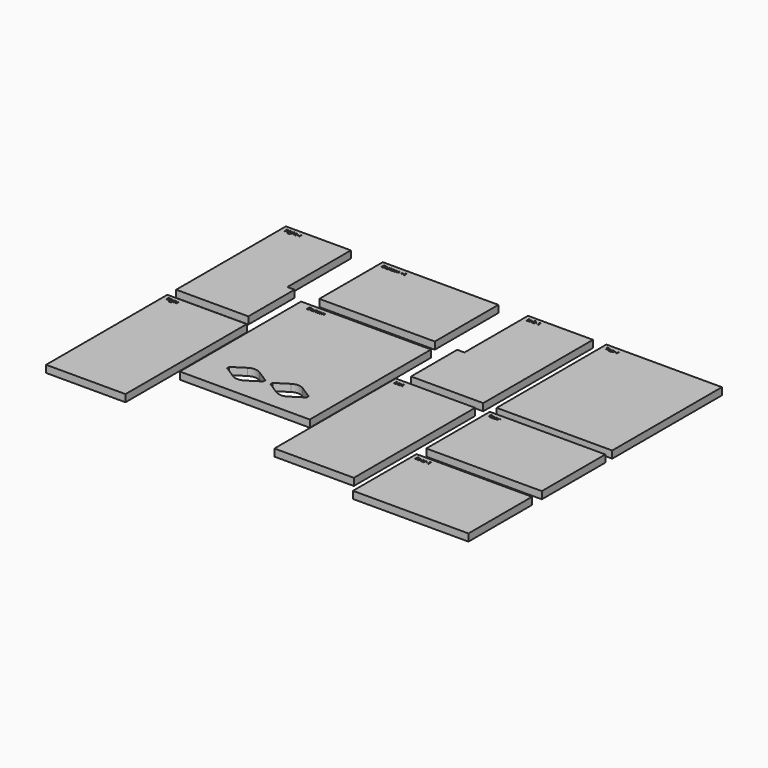
from build123d import *

# Parameters (mm, degrees)
F0_W     = 114.3
F0_H     = 133.35
F1_DEPTH = 6.35
F0_W_2   = 101.6
F0_H_2   = 69.85
F0_W_3   = 1.0569552951
F0_H_3   = 0.3272840712
F0_W_4   = 69.85
F0_W_5   = 0.3576009115
F0_H_4   = 2.359890408
F0_H_5   = 120.65


with BuildPart() as f1:
    # F0 (on Top) → F1 (new body)
    with BuildSketch(Plane.XY):
        with Locations((5.7540497959, -71.7852167927)):
            Rectangle(F0_W, F0_H)
        with BuildLine():
            ThreePointArc((-8.157172127, -121.0801036294), (-13.2959502041, -122.5852167927), (-18.4347282813, -121.0801036294))
            Line((-18.4347282813, -121.0801036294), (-29.1709502041, -114.2008217927))
            Line((-29.1709502041, -114.2008217927), (-29.1709502041, -111.9196117927))
            Line((-29.1709502041, -111.9196117927), (-18.4347282813, -105.0403299559))
            ThreePointArc((-18.4347282813, -105.0403299559), (-13.2959502041, -103.5352167927), (-8.157172127, -105.0403299559))
            Line((-8.157172127, -105.0403299559), (2.5790497959, -111.9196117927))
            Line((2.5790497959, -111.9196117927), (2.5790497959, -114.2008217927))
            Line((2.5790497959, -114.2008217927), (-8.157172127, -121.0801036294))
        make_face(mode=Mode.SUBTRACT)
        with BuildLine():
            ThreePointArc((29.942827873, -121.0801036294), (24.8040497959, -122.5852167927), (19.6652717187, -121.0801036294))
            Line((19.6652717187, -121.0801036294), (8.9290497959, -114.2008217927))
            Line((8.9290497959, -114.2008217927), (8.9290497959, -111.9196117927))
            Line((8.9290497959, -111.9196117927), (19.6652717187, -105.0403299559))
            ThreePointArc((19.6652717187, -105.0403299559), (24.8040497959, -103.5352167927), (29.942827873, -105.0403299559))
            Line((29.942827873, -105.0403299559), (40.6790497959, -111.9196117927))
            Line((40.6790497959, -111.9196117927), (40.6790497959, -114.2008217927))
            Line((40.6790497959, -114.2008217927), (29.942827873, -121.0801036294))
        make_face(mode=Mode.SUBTRACT)
        with BuildLine():
            Line((-41.4382462111, -11.4602167927), (-41.4382462111, -8.3120885375))
            Line((-41.4382462111, -8.3120885375), (-40.5487225566, -8.3120885375))
            add(Edge.make_bspline(
                [(-40.5487225566, -8.3120885375), (-39.9224041972, -8.3120885375), (-39.6423179342, -8.4995017319)],
                knots=[0, 0, 0, 1, 1, 1], degree=2))
            add(Edge.make_bspline(
                [(-39.6423179342, -8.4995017319), (-39.3622316711, -8.6869149264), (-39.3622316711, -9.0913691364)],
                knots=[0, 0, 0, 1, 1, 1], degree=2))
            add(Edge.make_bspline(
                [(-39.3622316711, -9.0913691364), (-39.3622316711, -9.371799909), (-39.5182944967, -9.5537009507)],
                knots=[0, 0, 0, 1, 1, 1], degree=2))
            add(Edge.make_bspline(
                [(-39.5182944967, -9.5537009507), (-39.6743573222, -9.7356019923), (-39.9740806295, -9.7893454819)],
                knots=[0, 0, 0, 1, 1, 1], degree=2))
            Line((-39.9740806295, -9.7893454819), (-39.9740806295, -9.8107050739))
            add(Edge.make_bspline(
                [(-39.9740806295, -9.8107050739), (-39.2568117493, -9.9333504732), (-39.2568117493, -10.5644919663)],
                knots=[0, 0, 0, 1, 1, 1], degree=2))
            add(Edge.make_bspline(
                [(-39.2568117493, -10.5644919663), (-39.2568117493, -10.9861716538), (-39.5420656555, -11.2231942232)],
                knots=[0, 0, 0, 1, 1, 1], degree=2))
            add(Edge.make_bspline(
                [(-39.5420656555, -11.2231942232), (-39.8273195618, -11.4602167927), (-40.3399497701, -11.4602167927)],
                knots=[0, 0, 0, 1, 1, 1], degree=2))
            Line((-40.3399497701, -11.4602167927), (-41.4382462111, -11.4602167927))
        make_face(mode=Mode.SUBTRACT)
        with BuildLine():
            add(Edge.make_bspline(
                [(-36.8896866408, -9.3866138196), (-36.5978870531, -9.7163094576), (-36.5978870531, -10.2778600218)],
                knots=[0, 0, 0, 1, 1, 1], degree=2))
            add(Edge.make_bspline(
                [(-36.5978870531, -10.2778600218), (-36.5978870531, -10.8552580253), (-36.8883086026, -11.1794415106)],
                knots=[0, 0, 0, 1, 1, 1], degree=2))
            add(Edge.make_bspline(
                [(-36.8883086026, -11.1794415106), (-37.1787301521, -11.5036249958), (-37.6913603604, -11.5036249958)],
                knots=[0, 0, 0, 1, 1, 1], degree=2))
            add(Edge.make_bspline(
                [(-37.6913603604, -11.5036249958), (-38.0083091451, -11.5036249958), (-38.2535999437, -11.3547968708)],
                knots=[0, 0, 0, 1, 1, 1], degree=2))
            add(Edge.make_bspline(
                [(-38.2535999437, -11.3547968708), (-38.4988907423, -11.2059687458), (-38.6325604472, -10.9282940496)],
                knots=[0, 0, 0, 1, 1, 1], degree=2))
            add(Edge.make_bspline(
                [(-38.6325604472, -10.9282940496), (-38.7662301521, -10.6506193534), (-38.7662301521, -10.2778600218)],
                knots=[0, 0, 0, 1, 1, 1], degree=2))
            add(Edge.make_bspline(
                [(-38.7662301521, -10.2778600218), (-38.7662301521, -9.7011510375), (-38.4775311503, -9.3790346095)],
                knots=[0, 0, 0, 1, 1, 1], degree=2))
            add(Edge.make_bspline(
                [(-38.4775311503, -9.3790346095), (-38.1888321486, -9.0569181816), (-37.6762019402, -9.0569181816)],
                knots=[0, 0, 0, 1, 1, 1], degree=2))
            add(Edge.make_bspline(
                [(-37.6762019402, -9.0569181816), (-37.1814862284, -9.0569181816), (-36.8896866408, -9.3866138196)],
                knots=[0, 0, 0, 1, 1, 1], degree=2))
        make_face(mode=Mode.SUBTRACT)
        with BuildLine():
            add(Edge.make_bspline(
                [(-35.4864992493, -11.0940031425), (-35.385213442, -11.2080358031), (-35.2088245531, -11.2080358031)],
                knots=[0, 0, 0, 1, 1, 1], degree=2))
            add(Edge.make_bspline(
                [(-35.2088245531, -11.2080358031), (-35.1137399177, -11.2080358031), (-35.0255454732, -11.1942554211)],
                knots=[0, 0, 0, 1, 1, 1], degree=2))
            add(Edge.make_bspline(
                [(-35.0255454732, -11.1942554211), (-34.9373510288, -11.1804750392), (-34.8856745965, -11.1653166191)],
                knots=[0, 0, 0, 1, 1, 1], degree=2))
            Line((-34.8856745965, -11.1653166191), (-34.8856745965, -11.4388572007))
            add(Edge.make_bspline(
                [(-34.8856745965, -11.4388572007), (-34.9435522007, -11.4664179645), (-35.0565513326, -11.4850214802)],
                knots=[0, 0, 0, 1, 1, 1], degree=2))
            add(Edge.make_bspline(
                [(-35.0565513326, -11.4850214802), (-35.1695504646, -11.5036249958), (-35.2605009854, -11.5036249958)],
                knots=[0, 0, 0, 1, 1, 1], degree=2))
            add(Edge.make_bspline(
                [(-35.2605009854, -11.5036249958), (-35.9446969489, -11.5036249958), (-35.9446969489, -10.782222001)],
                knots=[0, 0, 0, 1, 1, 1], degree=2))
            Line((-35.9446969489, -10.782222001), (-35.9446969489, -9.3780010809))
            Line((-35.9446969489, -9.3780010809), (-36.2830053257, -9.3780010809))
            Line((-36.2830053257, -9.3780010809), (-36.2830053257, -9.2057463066))
            Line((-36.2830053257, -9.2057463066), (-35.9446969489, -9.0569181816))
            Line((-35.9446969489, -9.0569181816), (-35.7944907857, -8.5532452215))
            Line((-35.7944907857, -8.5532452215), (-35.5877850566, -8.5532452215))
            Line((-35.5877850566, -8.5532452215), (-35.5877850566, -9.1003263847))
            Line((-35.5877850566, -9.1003263847), (-34.9029000739, -9.1003263847))
            Line((-34.9029000739, -9.1003263847), (-34.9029000739, -9.3780010809))
            Line((-34.9029000739, -9.3780010809), (-35.5877850566, -9.3780010809))
            Line((-35.5877850566, -9.3780010809), (-35.5877850566, -10.7670635809))
            add(Edge.make_bspline(
                [(-35.5877850566, -10.7670635809), (-35.5877850566, -10.9799704819), (-35.4864992493, -11.0940031425)],
                knots=[0, 0, 0, 1, 1, 1], degree=2))
        make_face(mode=Mode.SUBTRACT)
        with BuildLine():
            add(Edge.make_bspline(
                [(-33.9300051086, -11.0940031425), (-33.8287193014, -11.2080358031), (-33.6523304125, -11.2080358031)],
                knots=[0, 0, 0, 1, 1, 1], degree=2))
            add(Edge.make_bspline(
                [(-33.6523304125, -11.2080358031), (-33.5572457771, -11.2080358031), (-33.4690513326, -11.1942554211)],
                knots=[0, 0, 0, 1, 1, 1], degree=2))
            add(Edge.make_bspline(
                [(-33.4690513326, -11.1942554211), (-33.3808568882, -11.1804750392), (-33.3291804559, -11.1653166191)],
                knots=[0, 0, 0, 1, 1, 1], degree=2))
            Line((-33.3291804559, -11.1653166191), (-33.3291804559, -11.4388572007))
            add(Edge.make_bspline(
                [(-33.3291804559, -11.4388572007), (-33.38705806, -11.4664179645), (-33.500057192, -11.4850214802)],
                knots=[0, 0, 0, 1, 1, 1], degree=2))
            add(Edge.make_bspline(
                [(-33.500057192, -11.4850214802), (-33.6130563239, -11.5036249958), (-33.7040068448, -11.5036249958)],
                knots=[0, 0, 0, 1, 1, 1], degree=2))
            add(Edge.make_bspline(
                [(-33.7040068448, -11.5036249958), (-34.3882028083, -11.5036249958), (-34.3882028083, -10.782222001)],
                knots=[0, 0, 0, 1, 1, 1], degree=2))
            Line((-34.3882028083, -10.782222001), (-34.3882028083, -9.3780010809))
            Line((-34.3882028083, -9.3780010809), (-34.726511185, -9.3780010809))
            Line((-34.726511185, -9.3780010809), (-34.726511185, -9.2057463066))
            Line((-34.726511185, -9.2057463066), (-34.3882028083, -9.0569181816))
            Line((-34.3882028083, -9.0569181816), (-34.2379966451, -8.5532452215))
            Line((-34.2379966451, -8.5532452215), (-34.0312909159, -8.5532452215))
            Line((-34.0312909159, -8.5532452215), (-34.0312909159, -9.1003263847))
            Line((-34.0312909159, -9.1003263847), (-33.3464059333, -9.1003263847))
            Line((-33.3464059333, -9.1003263847), (-33.3464059333, -9.3780010809))
            Line((-33.3464059333, -9.3780010809), (-34.0312909159, -9.3780010809))
            Line((-34.0312909159, -9.3780010809), (-34.0312909159, -10.7670635809))
            add(Edge.make_bspline(
                [(-34.0312909159, -10.7670635809), (-34.0312909159, -10.9799704819), (-33.9300051086, -11.0940031425)],
                knots=[0, 0, 0, 1, 1, 1], degree=2))
        make_face(mode=Mode.SUBTRACT)
        with BuildLine():
            add(Edge.make_bspline(
                [(-31.1129505297, -9.3866138196), (-30.821150942, -9.7163094576), (-30.821150942, -10.2778600218)],
                knots=[0, 0, 0, 1, 1, 1], degree=2))
            add(Edge.make_bspline(
                [(-30.821150942, -10.2778600218), (-30.821150942, -10.8552580253), (-31.1115724915, -11.1794415106)],
                knots=[0, 0, 0, 1, 1, 1], degree=2))
            add(Edge.make_bspline(
                [(-31.1115724915, -11.1794415106), (-31.4019940409, -11.5036249958), (-31.9146242493, -11.5036249958)],
                knots=[0, 0, 0, 1, 1, 1], degree=2))
            add(Edge.make_bspline(
                [(-31.9146242493, -11.5036249958), (-32.231573034, -11.5036249958), (-32.4768638326, -11.3547968708)],
                knots=[0, 0, 0, 1, 1, 1], degree=2))
            add(Edge.make_bspline(
                [(-32.4768638326, -11.3547968708), (-32.7221546312, -11.2059687458), (-32.8558243361, -10.9282940496)],
                knots=[0, 0, 0, 1, 1, 1], degree=2))
            add(Edge.make_bspline(
                [(-32.8558243361, -10.9282940496), (-32.9894940409, -10.6506193534), (-32.9894940409, -10.2778600218)],
                knots=[0, 0, 0, 1, 1, 1], degree=2))
            add(Edge.make_bspline(
                [(-32.9894940409, -10.2778600218), (-32.9894940409, -9.7011510375), (-32.7007950392, -9.3790346095)],
                knots=[0, 0, 0, 1, 1, 1], degree=2))
            add(Edge.make_bspline(
                [(-32.7007950392, -9.3790346095), (-32.4120960375, -9.0569181816), (-31.8994658291, -9.0569181816)],
                knots=[0, 0, 0, 1, 1, 1], degree=2))
            add(Edge.make_bspline(
                [(-31.8994658291, -9.0569181816), (-31.4047501173, -9.0569181816), (-31.1129505297, -9.3866138196)],
                knots=[0, 0, 0, 1, 1, 1], degree=2))
        make_face(mode=Mode.SUBTRACT)
        with BuildLine():
            Line((-26.8289742927, -11.4602167927), (-27.185886185, -11.4602167927))
            Line((-27.185886185, -11.4602167927), (-27.185886185, -9.9250822441))
            add(Edge.make_bspline(
                [(-27.185886185, -9.9250822441), (-27.185886185, -9.6425844142), (-27.3064645271, -9.5016800088)],
                knots=[0, 0, 0, 1, 1, 1], degree=2))
            add(Edge.make_bspline(
                [(-27.3064645271, -9.5016800088), (-27.4270428691, -9.3607756034), (-27.6812909159, -9.3607756034)],
                knots=[0, 0, 0, 1, 1, 1], degree=2))
            add(Edge.make_bspline(
                [(-27.6812909159, -9.3607756034), (-28.014776159, -9.3607756034), (-28.17428408, -9.5523229125)],
                knots=[0, 0, 0, 1, 1, 1], degree=2))
            add(Edge.make_bspline(
                [(-28.17428408, -9.5523229125), (-28.333792001, -9.7438702215), (-28.333792001, -10.1421232597)],
                knots=[0, 0, 0, 1, 1, 1], degree=2))
            Line((-28.333792001, -10.1421232597), (-28.333792001, -11.4602167927))
            Line((-28.333792001, -11.4602167927), (-28.6913929125, -11.4602167927))
            Line((-28.6913929125, -11.4602167927), (-28.6913929125, -9.9250822441))
            add(Edge.make_bspline(
                [(-28.6913929125, -9.9250822441), (-28.6913929125, -9.6425844142), (-28.8119712545, -9.5016800088)],
                knots=[0, 0, 0, 1, 1, 1], degree=2))
            add(Edge.make_bspline(
                [(-28.8119712545, -9.5016800088), (-28.9325495965, -9.3607756034), (-29.1888647007, -9.3607756034)],
                knots=[0, 0, 0, 1, 1, 1], degree=2))
            add(Edge.make_bspline(
                [(-29.1888647007, -9.3607756034), (-29.524417001, -9.3607756034), (-29.6804798265, -9.5619691798)],
                knots=[0, 0, 0, 1, 1, 1], degree=2))
            add(Edge.make_bspline(
                [(-29.6804798265, -9.5619691798), (-29.8365426521, -9.7631627562), (-29.8365426521, -10.222049475)],
                knots=[0, 0, 0, 1, 1, 1], degree=2))
            Line((-29.8365426521, -10.222049475), (-29.8365426521, -11.4602167927))
            Line((-29.8365426521, -11.4602167927), (-30.1941435635, -11.4602167927))
            Line((-30.1941435635, -11.4602167927), (-30.1941435635, -9.1003263847))
            Line((-30.1941435635, -9.1003263847), (-29.9033775045, -9.1003263847))
            Line((-29.9033775045, -9.1003263847), (-29.8454999003, -9.4234763413))
            Line((-29.8454999003, -9.4234763413), (-29.8282744229, -9.4234763413))
            add(Edge.make_bspline(
                [(-29.8282744229, -9.4234763413), (-29.7269886156, -9.251221567), (-29.5426760071, -9.1540698743)],
                knots=[0, 0, 0, 1, 1, 1], degree=2))
            add(Edge.make_bspline(
                [(-29.5426760071, -9.1540698743), (-29.3583633986, -9.0569181816), (-29.1302980774, -9.0569181816)],
                knots=[0, 0, 0, 1, 1, 1], degree=2))
            add(Edge.make_bspline(
                [(-29.1302980774, -9.0569181816), (-28.5770157423, -9.0569181816), (-28.4068280253, -9.4579272961)],
                knots=[0, 0, 0, 1, 1, 1], degree=2))
            Line((-28.4068280253, -9.4579272961), (-28.3896025479, -9.4579272961))
            add(Edge.make_bspline(
                [(-28.3896025479, -9.4579272961), (-28.284182626, -9.272581159), (-28.0840225783, -9.1647496703)],
                knots=[0, 0, 0, 1, 1, 1], degree=2))
            add(Edge.make_bspline(
                [(-28.0840225783, -9.1647496703), (-27.8838625305, -9.0569181816), (-27.6275474264, -9.0569181816)],
                knots=[0, 0, 0, 1, 1, 1], degree=2))
            add(Edge.make_bspline(
                [(-27.6275474264, -9.0569181816), (-27.2272273309, -9.0569181816), (-27.0281008118, -9.2625903821)],
                knots=[0, 0, 0, 1, 1, 1], degree=2))
            add(Edge.make_bspline(
                [(-27.0281008118, -9.2625903821), (-26.8289742927, -9.4682625826), (-26.8289742927, -9.9209481295)],
                knots=[0, 0, 0, 1, 1, 1], degree=2))
            Line((-26.8289742927, -9.9209481295), (-26.8289742927, -11.4602167927))
        make_face(mode=Mode.SUBTRACT)
    extrude(amount=F1_DEPTH)


with BuildPart() as f1b:
    # F0 (on Top) → F1, piece 2 (new body)
    with BuildSketch(Plane.XY):
        with Locations((6.6755381465, 40.7469782948)):
            Rectangle(F0_W_2, F0_H_2)
        with BuildLine():
            add(Edge.make_bspline(
                [(-35.9681982901, 71.3955812679), (-35.6763987025, 71.0658856299), (-35.6763987025, 70.5043350657)],
                knots=[0, 0, 0, 1, 1, 1], degree=2))
            add(Edge.make_bspline(
                [(-35.6763987025, 70.5043350657), (-35.6763987025, 69.9269370622), (-35.9668202519, 69.602753577)],
                knots=[0, 0, 0, 1, 1, 1], degree=2))
            add(Edge.make_bspline(
                [(-35.9668202519, 69.602753577), (-36.2572418014, 69.2785700917), (-36.7698720098, 69.2785700917)],
                knots=[0, 0, 0, 1, 1, 1], degree=2))
            add(Edge.make_bspline(
                [(-36.7698720098, 69.2785700917), (-37.0868207945, 69.2785700917), (-37.3321115931, 69.4273982167)],
                knots=[0, 0, 0, 1, 1, 1], degree=2))
            add(Edge.make_bspline(
                [(-37.3321115931, 69.4273982167), (-37.5774023917, 69.5762263417), (-37.7110720966, 69.8539010379)],
                knots=[0, 0, 0, 1, 1, 1], degree=2))
            add(Edge.make_bspline(
                [(-37.7110720966, 69.8539010379), (-37.8447418014, 70.1315757341), (-37.8447418014, 70.5043350657)],
                knots=[0, 0, 0, 1, 1, 1], degree=2))
            add(Edge.make_bspline(
                [(-37.8447418014, 70.5043350657), (-37.8447418014, 71.0810440501), (-37.5560427997, 71.403160478)],
                knots=[0, 0, 0, 1, 1, 1], degree=2))
            add(Edge.make_bspline(
                [(-37.5560427997, 71.403160478), (-37.2673437979, 71.725276906), (-36.7547135896, 71.725276906)],
                knots=[0, 0, 0, 1, 1, 1], degree=2))
            add(Edge.make_bspline(
                [(-36.7547135896, 71.725276906), (-36.2599978778, 71.725276906), (-35.9681982901, 71.3955812679)],
                knots=[0, 0, 0, 1, 1, 1], degree=2))
        make_face(mode=Mode.SUBTRACT)
        with BuildLine():
            Line((-40.5167578604, 69.3219782948), (-40.5167578604, 72.4701065501))
            Line((-40.5167578604, 72.4701065501), (-39.6272342059, 72.4701065501))
            add(Edge.make_bspline(
                [(-39.6272342059, 72.4701065501), (-39.0009158466, 72.4701065501), (-38.7208295835, 72.2826933556)],
                knots=[0, 0, 0, 1, 1, 1], degree=2))
            add(Edge.make_bspline(
                [(-38.7208295835, 72.2826933556), (-38.4407433205, 72.0952801612), (-38.4407433205, 71.6908259511)],
                knots=[0, 0, 0, 1, 1, 1], degree=2))
            add(Edge.make_bspline(
                [(-38.4407433205, 71.6908259511), (-38.4407433205, 71.4103951785), (-38.596806146, 71.2284941369)],
                knots=[0, 0, 0, 1, 1, 1], degree=2))
            add(Edge.make_bspline(
                [(-38.596806146, 71.2284941369), (-38.7528689716, 71.0465930952), (-39.0525922789, 70.9928496056)],
                knots=[0, 0, 0, 1, 1, 1], degree=2))
            Line((-39.0525922789, 70.9928496056), (-39.0525922789, 70.9714900136))
            add(Edge.make_bspline(
                [(-39.0525922789, 70.9714900136), (-38.3353233986, 70.8488446143), (-38.3353233986, 70.2177031212)],
                knots=[0, 0, 0, 1, 1, 1], degree=2))
            add(Edge.make_bspline(
                [(-38.3353233986, 70.2177031212), (-38.3353233986, 69.7960234337), (-38.6205773049, 69.5590008643)],
                knots=[0, 0, 0, 1, 1, 1], degree=2))
            add(Edge.make_bspline(
                [(-38.6205773049, 69.5590008643), (-38.9058312111, 69.3219782948), (-39.4184614195, 69.3219782948)],
                knots=[0, 0, 0, 1, 1, 1], degree=2))
            Line((-39.4184614195, 69.3219782948), (-40.5167578604, 69.3219782948))
        make_face(mode=Mode.SUBTRACT)
        with BuildLine():
            add(Edge.make_bspline(
                [(-34.5650108986, 69.688191945), (-34.4637250914, 69.5741592844), (-34.2873362025, 69.5741592844)],
                knots=[0, 0, 0, 1, 1, 1], degree=2))
            add(Edge.make_bspline(
                [(-34.2873362025, 69.5741592844), (-34.192251567, 69.5741592844), (-34.1040571226, 69.5879396664)],
                knots=[0, 0, 0, 1, 1, 1], degree=2))
            add(Edge.make_bspline(
                [(-34.1040571226, 69.5879396664), (-34.0158626782, 69.6017200483), (-33.9641862459, 69.6168784685)],
                knots=[0, 0, 0, 1, 1, 1], degree=2))
            Line((-33.9641862459, 69.6168784685), (-33.9641862459, 69.3433378869))
            add(Edge.make_bspline(
                [(-33.9641862459, 69.3433378869), (-34.02206385, 69.315777123), (-34.135062982, 69.2971736073)],
                knots=[0, 0, 0, 1, 1, 1], degree=2))
            add(Edge.make_bspline(
                [(-34.135062982, 69.2971736073), (-34.2480621139, 69.2785700917), (-34.3390126348, 69.2785700917)],
                knots=[0, 0, 0, 1, 1, 1], degree=2))
            add(Edge.make_bspline(
                [(-34.3390126348, 69.2785700917), (-35.0232085983, 69.2785700917), (-35.0232085983, 69.9999730865)],
                knots=[0, 0, 0, 1, 1, 1], degree=2))
            Line((-35.0232085983, 69.9999730865), (-35.0232085983, 71.4041940067))
            Line((-35.0232085983, 71.4041940067), (-35.361516975, 71.4041940067))
            Line((-35.361516975, 71.4041940067), (-35.361516975, 71.576448781))
            Line((-35.361516975, 71.576448781), (-35.0232085983, 71.725276906))
            Line((-35.0232085983, 71.725276906), (-34.8730024351, 72.228949866))
            Line((-34.8730024351, 72.228949866), (-34.6662967059, 72.228949866))
            Line((-34.6662967059, 72.228949866), (-34.6662967059, 71.6818687028))
            Line((-34.6662967059, 71.6818687028), (-33.9814117233, 71.6818687028))
            Line((-33.9814117233, 71.6818687028), (-33.9814117233, 71.4041940067))
            Line((-33.9814117233, 71.4041940067), (-34.6662967059, 71.4041940067))
            Line((-34.6662967059, 71.4041940067), (-34.6662967059, 70.0151315067))
            add(Edge.make_bspline(
                [(-34.6662967059, 70.0151315067), (-34.6662967059, 69.8022246056), (-34.5650108986, 69.688191945)],
                knots=[0, 0, 0, 1, 1, 1], degree=2))
        make_face(mode=Mode.SUBTRACT)
        with BuildLine():
            add(Edge.make_bspline(
                [(-30.191462179, 71.3955812679), (-29.8996625914, 71.0658856299), (-29.8996625914, 70.5043350657)],
                knots=[0, 0, 0, 1, 1, 1], degree=2))
            add(Edge.make_bspline(
                [(-29.8996625914, 70.5043350657), (-29.8996625914, 69.9269370622), (-30.1900841408, 69.602753577)],
                knots=[0, 0, 0, 1, 1, 1], degree=2))
            add(Edge.make_bspline(
                [(-30.1900841408, 69.602753577), (-30.4805056903, 69.2785700917), (-30.9931358986, 69.2785700917)],
                knots=[0, 0, 0, 1, 1, 1], degree=2))
            add(Edge.make_bspline(
                [(-30.9931358986, 69.2785700917), (-31.3100846834, 69.2785700917), (-31.555375482, 69.4273982167)],
                knots=[0, 0, 0, 1, 1, 1], degree=2))
            add(Edge.make_bspline(
                [(-31.555375482, 69.4273982167), (-31.8006662806, 69.5762263417), (-31.9343359854, 69.8539010379)],
                knots=[0, 0, 0, 1, 1, 1], degree=2))
            add(Edge.make_bspline(
                [(-31.9343359854, 69.8539010379), (-32.0680056903, 70.1315757341), (-32.0680056903, 70.5043350657)],
                knots=[0, 0, 0, 1, 1, 1], degree=2))
            add(Edge.make_bspline(
                [(-32.0680056903, 70.5043350657), (-32.0680056903, 71.0810440501), (-31.7793066886, 71.403160478)],
                knots=[0, 0, 0, 1, 1, 1], degree=2))
            add(Edge.make_bspline(
                [(-31.7793066886, 71.403160478), (-31.4906076868, 71.725276906), (-30.9779774785, 71.725276906)],
                knots=[0, 0, 0, 1, 1, 1], degree=2))
            add(Edge.make_bspline(
                [(-30.9779774785, 71.725276906), (-30.4832617667, 71.725276906), (-30.191462179, 71.3955812679)],
                knots=[0, 0, 0, 1, 1, 1], degree=2))
        make_face(mode=Mode.SUBTRACT)
        with BuildLine():
            add(Edge.make_bspline(
                [(-33.008516758, 69.688191945), (-32.9072309507, 69.5741592844), (-32.7308420618, 69.5741592844)],
                knots=[0, 0, 0, 1, 1, 1], degree=2))
            add(Edge.make_bspline(
                [(-32.7308420618, 69.5741592844), (-32.6357574264, 69.5741592844), (-32.547562982, 69.5879396664)],
                knots=[0, 0, 0, 1, 1, 1], degree=2))
            add(Edge.make_bspline(
                [(-32.547562982, 69.5879396664), (-32.4593685375, 69.6017200483), (-32.4076921052, 69.6168784685)],
                knots=[0, 0, 0, 1, 1, 1], degree=2))
            Line((-32.4076921052, 69.6168784685), (-32.4076921052, 69.3433378869))
            add(Edge.make_bspline(
                [(-32.4076921052, 69.3433378869), (-32.4655697094, 69.315777123), (-32.5785688414, 69.2971736073)],
                knots=[0, 0, 0, 1, 1, 1], degree=2))
            add(Edge.make_bspline(
                [(-32.5785688414, 69.2971736073), (-32.6915679733, 69.2785700917), (-32.7825184941, 69.2785700917)],
                knots=[0, 0, 0, 1, 1, 1], degree=2))
            add(Edge.make_bspline(
                [(-32.7825184941, 69.2785700917), (-33.4667144577, 69.2785700917), (-33.4667144577, 69.9999730865)],
                knots=[0, 0, 0, 1, 1, 1], degree=2))
            Line((-33.4667144577, 69.9999730865), (-33.4667144577, 71.4041940067))
            Line((-33.4667144577, 71.4041940067), (-33.8050228344, 71.4041940067))
            Line((-33.8050228344, 71.4041940067), (-33.8050228344, 71.576448781))
            Line((-33.8050228344, 71.576448781), (-33.4667144577, 71.725276906))
            Line((-33.4667144577, 71.725276906), (-33.3165082945, 72.228949866))
            Line((-33.3165082945, 72.228949866), (-33.1098025653, 72.228949866))
            Line((-33.1098025653, 72.228949866), (-33.1098025653, 71.6818687028))
            Line((-33.1098025653, 71.6818687028), (-32.4249175827, 71.6818687028))
            Line((-32.4249175827, 71.6818687028), (-32.4249175827, 71.4041940067))
            Line((-32.4249175827, 71.4041940067), (-33.1098025653, 71.4041940067))
            Line((-33.1098025653, 71.4041940067), (-33.1098025653, 70.0151315067))
            add(Edge.make_bspline(
                [(-33.1098025653, 70.0151315067), (-33.1098025653, 69.8022246056), (-33.008516758, 69.688191945)],
                knots=[0, 0, 0, 1, 1, 1], degree=2))
        make_face(mode=Mode.SUBTRACT)
        with BuildLine():
            Line((-25.907485942, 69.3219782948), (-26.2643978344, 69.3219782948))
            Line((-26.2643978344, 69.3219782948), (-26.2643978344, 70.8571128435))
            add(Edge.make_bspline(
                [(-26.2643978344, 70.8571128435), (-26.2643978344, 71.1396106733), (-26.3849761764, 71.2805150787)],
                knots=[0, 0, 0, 1, 1, 1], degree=2))
            add(Edge.make_bspline(
                [(-26.3849761764, 71.2805150787), (-26.5055545184, 71.4214194841), (-26.7598025653, 71.4214194841)],
                knots=[0, 0, 0, 1, 1, 1], degree=2))
            add(Edge.make_bspline(
                [(-26.7598025653, 71.4214194841), (-27.0932878084, 71.4214194841), (-27.2527957294, 71.2298721751)],
                knots=[0, 0, 0, 1, 1, 1], degree=2))
            add(Edge.make_bspline(
                [(-27.2527957294, 71.2298721751), (-27.4123036504, 71.038324866), (-27.4123036504, 70.6400718278)],
                knots=[0, 0, 0, 1, 1, 1], degree=2))
            Line((-27.4123036504, 70.6400718278), (-27.4123036504, 69.3219782948))
            Line((-27.4123036504, 69.3219782948), (-27.7699045618, 69.3219782948))
            Line((-27.7699045618, 69.3219782948), (-27.7699045618, 70.8571128435))
            add(Edge.make_bspline(
                [(-27.7699045618, 70.8571128435), (-27.7699045618, 71.1396106733), (-27.8904829039, 71.2805150787)],
                knots=[0, 0, 0, 1, 1, 1], degree=2))
            add(Edge.make_bspline(
                [(-27.8904829039, 71.2805150787), (-28.0110612459, 71.4214194841), (-28.26737635, 71.4214194841)],
                knots=[0, 0, 0, 1, 1, 1], degree=2))
            add(Edge.make_bspline(
                [(-28.26737635, 71.4214194841), (-28.6029286504, 71.4214194841), (-28.7589914759, 71.2202259077)],
                knots=[0, 0, 0, 1, 1, 1], degree=2))
            add(Edge.make_bspline(
                [(-28.7589914759, 71.2202259077), (-28.9150543014, 71.0190323313), (-28.9150543014, 70.5601456126)],
                knots=[0, 0, 0, 1, 1, 1], degree=2))
            Line((-28.9150543014, 70.5601456126), (-28.9150543014, 69.3219782948))
            Line((-28.9150543014, 69.3219782948), (-29.2726552129, 69.3219782948))
            Line((-29.2726552129, 69.3219782948), (-29.2726552129, 71.6818687028))
            Line((-29.2726552129, 71.6818687028), (-28.9818891539, 71.6818687028))
            Line((-28.9818891539, 71.6818687028), (-28.9240115497, 71.3587187462))
            Line((-28.9240115497, 71.3587187462), (-28.9067860723, 71.3587187462))
            add(Edge.make_bspline(
                [(-28.9067860723, 71.3587187462), (-28.805500265, 71.5309735205), (-28.6211876565, 71.6281252133)],
                knots=[0, 0, 0, 1, 1, 1], degree=2))
            add(Edge.make_bspline(
                [(-28.6211876565, 71.6281252133), (-28.4368750479, 71.725276906), (-28.2088097268, 71.725276906)],
                knots=[0, 0, 0, 1, 1, 1], degree=2))
            add(Edge.make_bspline(
                [(-28.2088097268, 71.725276906), (-27.6555273917, 71.725276906), (-27.4853396747, 71.3242677914)],
                knots=[0, 0, 0, 1, 1, 1], degree=2))
            Line((-27.4853396747, 71.3242677914), (-27.4681141973, 71.3242677914))
            add(Edge.make_bspline(
                [(-27.4681141973, 71.3242677914), (-27.3626942754, 71.5096139285), (-27.1625342276, 71.6174454172)],
                knots=[0, 0, 0, 1, 1, 1], degree=2))
            add(Edge.make_bspline(
                [(-27.1625342276, 71.6174454172), (-26.9623741799, 71.725276906), (-26.7060590757, 71.725276906)],
                knots=[0, 0, 0, 1, 1, 1], degree=2))
            add(Edge.make_bspline(
                [(-26.7060590757, 71.725276906), (-26.3057389802, 71.725276906), (-26.1066124611, 71.5196047054)],
                knots=[0, 0, 0, 1, 1, 1], degree=2))
            add(Edge.make_bspline(
                [(-26.1066124611, 71.5196047054), (-25.907485942, 71.3139325049), (-25.907485942, 70.861246958)],
                knots=[0, 0, 0, 1, 1, 1], degree=2))
            Line((-25.907485942, 70.861246958), (-25.907485942, 69.3219782948))
        make_face(mode=Mode.SUBTRACT)
        Polygon((-22.9977582945, 71.9464520362), (-22.9977582945, 71.0252335032), (-22.1109907164, 71.0252335032), (-22.1109907164, 70.7282662723), (-22.9977582945, 70.7282662723), (-22.9977582945, 69.8104928348), (-23.2974816018, 69.8104928348), (-23.2974816018, 70.7282662723), (-24.1801150653, 70.7282662723), (-24.1801150653, 71.0252335032), (-23.2974816018, 71.0252335032), (-23.2974816018, 71.9464520362), align=None, mode=Mode.SUBTRACT)
        with BuildLine():
            Line((-20.343656732, 72.4701065501), (-20.343656732, 69.3219782948))
            Line((-20.343656732, 69.3219782948), (-20.6923003952, 69.3219782948))
            Line((-20.6923003952, 69.3219782948), (-20.6923003952, 71.5654244754))
            add(Edge.make_bspline(
                [(-20.6923003952, 71.5654244754), (-20.6923003952, 71.845855248), (-20.6750749177, 72.0952801612)],
                knots=[0, 0, 0, 1, 1, 1], degree=2))
            add(Edge.make_bspline(
                [(-20.6750749177, 72.0952801612), (-20.7198611591, 72.0498049008), (-20.7760162155, 72.0005400353)],
                knots=[0, 0, 0, 1, 1, 1], degree=2))
            add(Edge.make_bspline(
                [(-20.7760162155, 72.0005400353), (-20.8321712719, 71.9512751698), (-21.2883019143, 71.5805828955)],
                knots=[0, 0, 0, 1, 1, 1], degree=2))
            Line((-21.2883019143, 71.5805828955), (-21.477782166, 71.8258736942))
            Line((-21.477782166, 71.8258736942), (-20.6447580775, 72.4701065501))
            Line((-20.6447580775, 72.4701065501), (-20.343656732, 72.4701065501))
        make_face(mode=Mode.SUBTRACT)
    extrude(amount=F1_DEPTH)


with BuildPart() as f1c:
    # F0 (on Top) → F1, piece 3 (new body)
    with BuildSketch(Plane.XY):
        Polygon((140.7129478097, 75.6719782948), (83.5629478097, 75.6719782948), (83.5629478097, 5.8219782948), (77.2129478097, 5.8219782948), (77.2129478097, -44.9780217052), (83.5629478097, -44.9780217052), (140.7129478097, -44.9780217052), align=None)
        Polygon((88.9255834434, 69.3219782948), (87.1706518028, 69.3219782948), (87.1706518028, 72.4701065501), (87.5365209434, 72.4701065501), (87.5365209434, 69.6533964806), (88.9255834434, 69.6533964806), align=None, mode=Mode.SUBTRACT)
        with BuildLine():
            add(Edge.make_bspline(
                [(90.8107396934, 69.3143990848), (90.6419300146, 69.2785700917), (90.4028403878, 69.2785700917)],
                knots=[0, 0, 0, 1, 1, 1], degree=2))
            add(Edge.make_bspline(
                [(90.4028403878, 69.2785700917), (89.879874893, 69.2785700917), (89.5770509998, 69.5975859337)],
                knots=[0, 0, 0, 1, 1, 1], degree=2))
            add(Edge.make_bspline(
                [(89.5770509998, 69.5975859337), (89.2742271066, 69.9166017758), (89.2742271066, 70.4822864546)],
                knots=[0, 0, 0, 1, 1, 1], degree=2))
            add(Edge.make_bspline(
                [(89.2742271066, 70.4822864546), (89.2742271066, 71.0534832862), (89.5553468982, 71.3893800961)],
                knots=[0, 0, 0, 1, 1, 1], degree=2))
            add(Edge.make_bspline(
                [(89.5553468982, 71.3893800961), (89.8364666899, 71.725276906), (90.3105118288, 71.725276906)],
                knots=[0, 0, 0, 1, 1, 1], degree=2))
            add(Edge.make_bspline(
                [(90.3105118288, 71.725276906), (90.7535511083, 71.725276906), (91.0119332698, 71.4334773183)],
                knots=[0, 0, 0, 1, 1, 1], degree=2))
            add(Edge.make_bspline(
                [(91.0119332698, 71.4334773183), (91.2703154312, 71.1416777306), (91.2703154312, 70.6634984771)],
                knots=[0, 0, 0, 1, 1, 1], degree=2))
            Line((91.2703154312, 70.6634984771), (91.2703154312, 70.4375002133))
            Line((91.2703154312, 70.4375002133), (89.6449193809, 70.4375002133))
            add(Edge.make_bspline(
                [(89.6449193809, 70.4375002133), (89.6559436864, 70.0220216976), (89.8550702055, 69.8067032297)],
                knots=[0, 0, 0, 1, 1, 1], degree=2))
            add(Edge.make_bspline(
                [(89.8550702055, 69.8067032297), (90.0541967246, 69.5913847619), (90.4159317507, 69.5913847619)],
                knots=[0, 0, 0, 1, 1, 1], degree=2))
            add(Edge.make_bspline(
                [(90.4159317507, 69.5913847619), (90.7969593114, 69.5913847619), (91.1690296239, 69.7505481733)],
                knots=[0, 0, 0, 1, 1, 1], degree=2))
            Line((91.1690296239, 69.7505481733), (91.1690296239, 69.4315323313))
            add(Edge.make_bspline(
                [(91.1690296239, 69.4315323313), (90.9795493722, 69.3502280778), (90.8107396934, 69.3143990848)],
                knots=[0, 0, 0, 1, 1, 1], degree=2))
        make_face(mode=Mode.SUBTRACT)
        with BuildLine():
            Line((92.9439428184, 71.6818687028), (92.9439428184, 71.4041940067))
            Line((92.9439428184, 71.4041940067), (92.3431181656, 71.4041940067))
            Line((92.3431181656, 71.4041940067), (92.3431181656, 69.3219782948))
            Line((92.3431181656, 69.3219782948), (91.9855172541, 69.3219782948))
            Line((91.9855172541, 69.3219782948), (91.9855172541, 71.4041940067))
            Line((91.9855172541, 71.4041940067), (91.5638375666, 71.4041940067))
            Line((91.5638375666, 71.4041940067), (91.5638375666, 71.5654244754))
            Line((91.5638375666, 71.5654244754), (91.9855172541, 71.6949600657))
            Line((91.9855172541, 71.6949600657), (91.9855172541, 71.8258736942))
            add(Edge.make_bspline(
                [(91.9855172541, 71.8258736942), (91.9855172541, 72.6961048139), (92.7455053184, 72.6961048139)],
                knots=[0, 0, 0, 1, 1, 1], degree=2))
            add(Edge.make_bspline(
                [(92.7455053184, 72.6961048139), (92.9329185128, 72.6961048139), (93.1850995024, 72.6210017323)],
                knots=[0, 0, 0, 1, 1, 1], degree=2))
            Line((93.1850995024, 72.6210017323), (93.0920819243, 72.3343697879))
            add(Edge.make_bspline(
                [(93.0920819243, 72.3343697879), (92.8853761951, 72.4012046403), (92.7393041465, 72.4012046403)],
                knots=[0, 0, 0, 1, 1, 1], degree=2))
            add(Edge.make_bspline(
                [(92.7393041465, 72.4012046403), (92.5367325319, 72.4012046403), (92.4399253488, 72.2665014068)],
                knots=[0, 0, 0, 1, 1, 1], degree=2))
            add(Edge.make_bspline(
                [(92.4399253488, 72.2665014068), (92.3431181656, 72.1317981733), (92.3431181656, 71.8348309424)],
                knots=[0, 0, 0, 1, 1, 1], degree=2))
            Line((92.3431181656, 71.8348309424), (92.3431181656, 71.6818687028))
            Line((92.3431181656, 71.6818687028), (92.9439428184, 71.6818687028))
        make_face(mode=Mode.SUBTRACT)
        with BuildLine():
            add(Edge.make_bspline(
                [(93.8589601795, 69.688191945), (93.9602459868, 69.5741592844), (94.1366348757, 69.5741592844)],
                knots=[0, 0, 0, 1, 1, 1], degree=2))
            add(Edge.make_bspline(
                [(94.1366348757, 69.5741592844), (94.2317195111, 69.5741592844), (94.3199139555, 69.5879396664)],
                knots=[0, 0, 0, 1, 1, 1], degree=2))
            add(Edge.make_bspline(
                [(94.3199139555, 69.5879396664), (94.4081084, 69.6017200483), (94.4597848323, 69.6168784685)],
                knots=[0, 0, 0, 1, 1, 1], degree=2))
            Line((94.4597848323, 69.6168784685), (94.4597848323, 69.3433378869))
            add(Edge.make_bspline(
                [(94.4597848323, 69.3433378869), (94.4019072281, 69.315777123), (94.2889080962, 69.2971736073)],
                knots=[0, 0, 0, 1, 1, 1], degree=2))
            add(Edge.make_bspline(
                [(94.2889080962, 69.2971736073), (94.1759089642, 69.2785700917), (94.0849584434, 69.2785700917)],
                knots=[0, 0, 0, 1, 1, 1], degree=2))
            add(Edge.make_bspline(
                [(94.0849584434, 69.2785700917), (93.4007624798, 69.2785700917), (93.4007624798, 69.9999730865)],
                knots=[0, 0, 0, 1, 1, 1], degree=2))
            Line((93.4007624798, 69.9999730865), (93.4007624798, 71.4041940067))
            Line((93.4007624798, 71.4041940067), (93.0624541031, 71.4041940067))
            Line((93.0624541031, 71.4041940067), (93.0624541031, 71.576448781))
            Line((93.0624541031, 71.576448781), (93.4007624798, 71.725276906))
            Line((93.4007624798, 71.725276906), (93.550968643, 72.228949866))
            Line((93.550968643, 72.228949866), (93.7576743722, 72.228949866))
            Line((93.7576743722, 72.228949866), (93.7576743722, 71.6818687028))
            Line((93.7576743722, 71.6818687028), (94.4425593548, 71.6818687028))
            Line((94.4425593548, 71.6818687028), (94.4425593548, 71.4041940067))
            Line((94.4425593548, 71.4041940067), (93.7576743722, 71.4041940067))
            Line((93.7576743722, 71.4041940067), (93.7576743722, 70.0151315067))
            add(Edge.make_bspline(
                [(93.7576743722, 70.0151315067), (93.7576743722, 69.8022246056), (93.8589601795, 69.688191945)],
                knots=[0, 0, 0, 1, 1, 1], degree=2))
        make_face(mode=Mode.SUBTRACT)
        with Locations((95.2618030614, 70.5039905561)):
            Rectangle(F0_W_3, F0_H_3, mode=Mode.SUBTRACT)
        with BuildLine():
            Line((97.5100723757, 72.4701065501), (97.5100723757, 69.3219782948))
            Line((97.5100723757, 69.3219782948), (97.1614287125, 69.3219782948))
            Line((97.1614287125, 69.3219782948), (97.1614287125, 71.5654244754))
            add(Edge.make_bspline(
                [(97.1614287125, 71.5654244754), (97.1614287125, 71.845855248), (97.1786541899, 72.0952801612)],
                knots=[0, 0, 0, 1, 1, 1], degree=2))
            add(Edge.make_bspline(
                [(97.1786541899, 72.0952801612), (97.1338679486, 72.0498049008), (97.0777128922, 72.0005400353)],
                knots=[0, 0, 0, 1, 1, 1], degree=2))
            add(Edge.make_bspline(
                [(97.0777128922, 72.0005400353), (97.0215578357, 71.9512751698), (96.5654271934, 71.5805828955)],
                knots=[0, 0, 0, 1, 1, 1], degree=2))
            Line((96.5654271934, 71.5805828955), (96.3759469416, 71.8258736942))
            Line((96.3759469416, 71.8258736942), (97.2089710302, 72.4701065501))
            Line((97.2089710302, 72.4701065501), (97.5100723757, 72.4701065501))
        make_face(mode=Mode.SUBTRACT)
    extrude(amount=F1_DEPTH)


with BuildPart() as f1d:
    # F0 (on Top) → F1, piece 4 (new body)
    with BuildSketch(Plane.XY):
        with Locations((105.7879478097, -120.5828935981)):
            Rectangle(F0_W_4, F0_H)
        with BuildLine():
            add(Edge.make_bspline(
                [(78.1107396934, -60.2654728081), (77.9419300146, -60.3013018012), (77.7028403878, -60.3013018012)],
                knots=[0, 0, 0, 1, 1, 1], degree=2))
            add(Edge.make_bspline(
                [(77.7028403878, -60.3013018012), (77.179874893, -60.3013018012), (76.8770509998, -59.9822859592)],
                knots=[0, 0, 0, 1, 1, 1], degree=2))
            add(Edge.make_bspline(
                [(76.8770509998, -59.9822859592), (76.5742271066, -59.6632701172), (76.5742271066, -59.0975854384)],
                knots=[0, 0, 0, 1, 1, 1], degree=2))
            add(Edge.make_bspline(
                [(76.5742271066, -59.0975854384), (76.5742271066, -58.5263886068), (76.8553468982, -58.1904917969)],
                knots=[0, 0, 0, 1, 1, 1], degree=2))
            add(Edge.make_bspline(
                [(76.8553468982, -58.1904917969), (77.1364666899, -57.854594987), (77.6105118288, -57.854594987)],
                knots=[0, 0, 0, 1, 1, 1], degree=2))
            add(Edge.make_bspline(
                [(77.6105118288, -57.854594987), (78.0535511083, -57.854594987), (78.3119332698, -58.1463945746)],
                knots=[0, 0, 0, 1, 1, 1], degree=2))
            add(Edge.make_bspline(
                [(78.3119332698, -58.1463945746), (78.5703154312, -58.4381941623), (78.5703154312, -58.9163734158)],
                knots=[0, 0, 0, 1, 1, 1], degree=2))
            Line((78.5703154312, -58.9163734158), (78.5703154312, -59.1423716797))
            Line((78.5703154312, -59.1423716797), (76.9449193809, -59.1423716797))
            add(Edge.make_bspline(
                [(76.9449193809, -59.1423716797), (76.9559436864, -59.5578501953), (77.1550702055, -59.7731686632)],
                knots=[0, 0, 0, 1, 1, 1], degree=2))
            add(Edge.make_bspline(
                [(77.1550702055, -59.7731686632), (77.3541967246, -59.9884871311), (77.7159317507, -59.9884871311)],
                knots=[0, 0, 0, 1, 1, 1], degree=2))
            add(Edge.make_bspline(
                [(77.7159317507, -59.9884871311), (78.0969593114, -59.9884871311), (78.4690296239, -59.8293237196)],
                knots=[0, 0, 0, 1, 1, 1], degree=2))
            Line((78.4690296239, -59.8293237196), (78.4690296239, -60.1483395616))
            add(Edge.make_bspline(
                [(78.4690296239, -60.1483395616), (78.2795493722, -60.2296438151), (78.1107396934, -60.2654728081)],
                knots=[0, 0, 0, 1, 1, 1], degree=2))
        make_face(mode=Mode.SUBTRACT)
        Polygon((76.2255834434, -60.2578935981), (74.4706518028, -60.2578935981), (74.4706518028, -57.1097653429), (74.8365209434, -57.1097653429), (74.8365209434, -59.9264754123), (76.2255834434, -59.9264754123), align=None, mode=Mode.SUBTRACT)
        with BuildLine():
            Line((80.2439428184, -57.8980031901), (80.2439428184, -58.1756778863))
            Line((80.2439428184, -58.1756778863), (79.6431181656, -58.1756778863))
            Line((79.6431181656, -58.1756778863), (79.6431181656, -60.2578935981))
            Line((79.6431181656, -60.2578935981), (79.2855172541, -60.2578935981))
            Line((79.2855172541, -60.2578935981), (79.2855172541, -58.1756778863))
            Line((79.2855172541, -58.1756778863), (78.8638375666, -58.1756778863))
            Line((78.8638375666, -58.1756778863), (78.8638375666, -58.0144474175))
            Line((78.8638375666, -58.0144474175), (79.2855172541, -57.8849118272))
            Line((79.2855172541, -57.8849118272), (79.2855172541, -57.7539981988))
            add(Edge.make_bspline(
                [(79.2855172541, -57.7539981988), (79.2855172541, -56.883767079), (80.0455053184, -56.883767079)],
                knots=[0, 0, 0, 1, 1, 1], degree=2))
            add(Edge.make_bspline(
                [(80.0455053184, -56.883767079), (80.2329185128, -56.883767079), (80.4850995024, -56.9588701606)],
                knots=[0, 0, 0, 1, 1, 1], degree=2))
            Line((80.4850995024, -56.9588701606), (80.3920819243, -57.245502105))
            add(Edge.make_bspline(
                [(80.3920819243, -57.245502105), (80.1853761951, -57.1786672526), (80.0393041465, -57.1786672526)],
                knots=[0, 0, 0, 1, 1, 1], degree=2))
            add(Edge.make_bspline(
                [(80.0393041465, -57.1786672526), (79.8367325319, -57.1786672526), (79.7399253488, -57.3133704861)],
                knots=[0, 0, 0, 1, 1, 1], degree=2))
            add(Edge.make_bspline(
                [(79.7399253488, -57.3133704861), (79.6431181656, -57.4480737196), (79.6431181656, -57.7450409505)],
                knots=[0, 0, 0, 1, 1, 1], degree=2))
            Line((79.6431181656, -57.7450409505), (79.6431181656, -57.8980031901))
            Line((79.6431181656, -57.8980031901), (80.2439428184, -57.8980031901))
        make_face(mode=Mode.SUBTRACT)
        with BuildLine():
            add(Edge.make_bspline(
                [(81.1589601795, -59.8916799479), (81.2602459868, -60.0057126085), (81.4366348757, -60.0057126085)],
                knots=[0, 0, 0, 1, 1, 1], degree=2))
            add(Edge.make_bspline(
                [(81.4366348757, -60.0057126085), (81.5317195111, -60.0057126085), (81.6199139555, -59.9919322266)],
                knots=[0, 0, 0, 1, 1, 1], degree=2))
            add(Edge.make_bspline(
                [(81.6199139555, -59.9919322266), (81.7081084, -59.9781518446), (81.7597848323, -59.9629934245)],
                knots=[0, 0, 0, 1, 1, 1], degree=2))
            Line((81.7597848323, -59.9629934245), (81.7597848323, -60.2365340061))
            add(Edge.make_bspline(
                [(81.7597848323, -60.2365340061), (81.7019072281, -60.26409477), (81.5889080962, -60.2826982856)],
                knots=[0, 0, 0, 1, 1, 1], degree=2))
            add(Edge.make_bspline(
                [(81.5889080962, -60.2826982856), (81.4759089642, -60.3013018012), (81.3849584434, -60.3013018012)],
                knots=[0, 0, 0, 1, 1, 1], degree=2))
            add(Edge.make_bspline(
                [(81.3849584434, -60.3013018012), (80.7007624798, -60.3013018012), (80.7007624798, -59.5798988064)],
                knots=[0, 0, 0, 1, 1, 1], degree=2))
            Line((80.7007624798, -59.5798988064), (80.7007624798, -58.1756778863))
            Line((80.7007624798, -58.1756778863), (80.3624541031, -58.1756778863))
            Line((80.3624541031, -58.1756778863), (80.3624541031, -58.003423112))
            Line((80.3624541031, -58.003423112), (80.7007624798, -57.854594987))
            Line((80.7007624798, -57.854594987), (80.850968643, -57.3509220269))
            Line((80.850968643, -57.3509220269), (81.0576743722, -57.3509220269))
            Line((81.0576743722, -57.3509220269), (81.0576743722, -57.8980031901))
            Line((81.0576743722, -57.8980031901), (81.7425593548, -57.8980031901))
            Line((81.7425593548, -57.8980031901), (81.7425593548, -58.1756778863))
            Line((81.7425593548, -58.1756778863), (81.0576743722, -58.1756778863))
            Line((81.0576743722, -58.1756778863), (81.0576743722, -59.5647403863))
            add(Edge.make_bspline(
                [(81.0576743722, -59.5647403863), (81.0576743722, -59.7776472873), (81.1589601795, -59.8916799479)],
                knots=[0, 0, 0, 1, 1, 1], degree=2))
        make_face(mode=Mode.SUBTRACT)
    extrude(amount=F1_DEPTH)


with BuildPart() as f1e:
    # F0 (on Top) → F1, piece 5 (new body)
    with BuildSketch(Plane.XY):
        Polygon((-72.2440544128, 75.6719782948), (-129.3940544128, 75.6719782948), (-129.3940544128, -44.9780217052), (-72.2440544128, -44.9780217052), (-65.8940544128, -44.9780217052), (-65.8940544128, 5.8219782948), (-72.2440544128, 5.8219782948), align=None)
        with BuildLine():
            Line((-124.7631570604, 70.6311145796), (-125.4204812792, 70.6311145796))
            Line((-125.4204812792, 70.6311145796), (-125.4204812792, 69.3219782948))
            Line((-125.4204812792, 69.3219782948), (-125.7863504198, 69.3219782948))
            Line((-125.7863504198, 69.3219782948), (-125.7863504198, 72.4701065501))
            Line((-125.7863504198, 72.4701065501), (-124.923009491, 72.4701065501))
            add(Edge.make_bspline(
                [(-124.923009491, 72.4701065501), (-124.3435444302, 72.4701065501), (-124.0669032627, 72.2482424008)],
                knots=[0, 0, 0, 1, 1, 1], degree=2))
            add(Edge.make_bspline(
                [(-124.0669032627, 72.2482424008), (-123.7902620951, 72.0263782514), (-123.7902620951, 71.5805828955)],
                knots=[0, 0, 0, 1, 1, 1], degree=2))
            add(Edge.make_bspline(
                [(-123.7902620951, 71.5805828955), (-123.7902620951, 70.9563315935), (-124.4234706455, 70.7365345014)],
                knots=[0, 0, 0, 1, 1, 1], degree=2))
            Line((-124.4234706455, 70.7365345014), (-123.5683979458, 69.3219782948))
            Line((-123.5683979458, 69.3219782948), (-124.0011019389, 69.3219782948))
            Line((-124.0011019389, 69.3219782948), (-124.7631570604, 70.6311145796))
        make_face(mode=Mode.SUBTRACT)
        with Locations((-122.935533905, 70.5019234988)):
            Rectangle(F0_W_5, F0_H_4, mode=Mode.SUBTRACT)
        with BuildLine():
            Line((-120.883290524, 71.6818687028), (-120.0674919128, 71.6818687028))
            Line((-120.0674919128, 71.6818687028), (-120.0674919128, 71.4558704389))
            Line((-120.0674919128, 71.4558704389), (-120.5043300205, 71.4041940067))
            add(Edge.make_bspline(
                [(-120.5043300205, 71.4041940067), (-120.444385359, 71.3290909251), (-120.3968430413, 71.2071345448)],
                knots=[0, 0, 0, 1, 1, 1], degree=2))
            add(Edge.make_bspline(
                [(-120.3968430413, 71.2071345448), (-120.3493007236, 71.0851781646), (-120.3493007236, 70.9329049442)],
                knots=[0, 0, 0, 1, 1, 1], degree=2))
            add(Edge.make_bspline(
                [(-120.3493007236, 70.9329049442), (-120.3493007236, 70.5856393192), (-120.5863232931, 70.37893359)],
                knots=[0, 0, 0, 1, 1, 1], degree=2))
            add(Edge.make_bspline(
                [(-120.5863232931, 70.37893359), (-120.8233458625, 70.1722278608), (-121.2367573208, 70.1722278608)],
                knots=[0, 0, 0, 1, 1, 1], degree=2))
            add(Edge.make_bspline(
                [(-121.2367573208, 70.1722278608), (-121.3421772427, 70.1722278608), (-121.4345058017, 70.1894533383)],
                knots=[0, 0, 0, 1, 1, 1], degree=2))
            add(Edge.make_bspline(
                [(-121.4345058017, 70.1894533383), (-121.6625711229, 70.0688749962), (-121.6625711229, 69.8862849355)],
                knots=[0, 0, 0, 1, 1, 1], degree=2))
            add(Edge.make_bspline(
                [(-121.6625711229, 69.8862849355), (-121.6625711229, 69.7891332428), (-121.5829894172, 69.7429689633)],
                knots=[0, 0, 0, 1, 1, 1], degree=2))
            add(Edge.make_bspline(
                [(-121.5829894172, 69.7429689633), (-121.5034077115, 69.6968046837), (-121.3097933451, 69.6968046837)],
                knots=[0, 0, 0, 1, 1, 1], degree=2))
            Line((-121.3097933451, 69.6968046837), (-120.8922477722, 69.6968046837))
            add(Edge.make_bspline(
                [(-120.8922477722, 69.6968046837), (-120.5084641351, 69.6968046837), (-120.3031364441, 69.5352297054)],
                knots=[0, 0, 0, 1, 1, 1], degree=2))
            add(Edge.make_bspline(
                [(-120.3031364441, 69.5352297054), (-120.0978087531, 69.3736547271), (-120.0978087531, 69.0656631907)],
                knots=[0, 0, 0, 1, 1, 1], degree=2))
            add(Edge.make_bspline(
                [(-120.0978087531, 69.0656631907), (-120.0978087531, 68.6736113244), (-120.4120014615, 68.4679391238)],
                knots=[0, 0, 0, 1, 1, 1], degree=2))
            add(Edge.make_bspline(
                [(-120.4120014615, 68.4679391238), (-120.7261941698, 68.2622669233), (-121.3290858799, 68.2622669233)],
                knots=[0, 0, 0, 1, 1, 1], degree=2))
            add(Edge.make_bspline(
                [(-121.3290858799, 68.2622669233), (-121.7921067132, 68.2622669233), (-122.0429096646, 68.4345216976)],
                knots=[0, 0, 0, 1, 1, 1], degree=2))
            add(Edge.make_bspline(
                [(-122.0429096646, 68.4345216976), (-122.293712616, 68.6067764719), (-122.293712616, 68.9216581994)],
                knots=[0, 0, 0, 1, 1, 1], degree=2))
            add(Edge.make_bspline(
                [(-122.293712616, 68.9216581994), (-122.293712616, 69.1366321577), (-122.1559087965, 69.2940730214)],
                knots=[0, 0, 0, 1, 1, 1], degree=2))
            add(Edge.make_bspline(
                [(-122.1559087965, 69.2940730214), (-122.0181049771, 69.4515138851), (-121.7686800639, 69.507324432)],
                knots=[0, 0, 0, 1, 1, 1], degree=2))
            add(Edge.make_bspline(
                [(-121.7686800639, 69.507324432), (-121.8589415656, 69.5479765587), (-121.9202642653, 69.6341039459)],
                knots=[0, 0, 0, 1, 1, 1], degree=2))
            add(Edge.make_bspline(
                [(-121.9202642653, 69.6341039459), (-121.9815869649, 69.720231333), (-121.9815869649, 69.8346085032)],
                knots=[0, 0, 0, 1, 1, 1], degree=2))
            add(Edge.make_bspline(
                [(-121.9815869649, 69.8346085032), (-121.9815869649, 69.9634550744), (-121.9126850552, 70.0606067671)],
                knots=[0, 0, 0, 1, 1, 1], degree=2))
            add(Edge.make_bspline(
                [(-121.9126850552, 70.0606067671), (-121.8437831455, 70.1577584598), (-121.6949550205, 70.2480199615)],
                knots=[0, 0, 0, 1, 1, 1], degree=2))
            add(Edge.make_bspline(
                [(-121.6949550205, 70.2480199615), (-121.8782341003, 70.3231230431), (-121.9933002896, 70.5039905561)],
                knots=[0, 0, 0, 1, 1, 1], degree=2))
            add(Edge.make_bspline(
                [(-121.9933002896, 70.5039905561), (-122.1083664788, 70.6848580692), (-122.1083664788, 70.917746524)],
                knots=[0, 0, 0, 1, 1, 1], degree=2))
            add(Edge.make_bspline(
                [(-122.1083664788, 70.917746524), (-122.1083664788, 71.3049752567), (-121.8758225335, 71.5151260813)],
                knots=[0, 0, 0, 1, 1, 1], degree=2))
            add(Edge.make_bspline(
                [(-121.8758225335, 71.5151260813), (-121.6432785882, 71.725276906), (-121.2174647861, 71.725276906)],
                knots=[0, 0, 0, 1, 1, 1], degree=2))
            add(Edge.make_bspline(
                [(-121.2174647861, 71.725276906), (-121.032118649, 71.725276906), (-120.883290524, 71.6818687028)],
                knots=[0, 0, 0, 1, 1, 1], degree=2))
        make_face(mode=Mode.SUBTRACT)
        with BuildLine():
            Line((-117.6104498121, 69.3219782948), (-117.9680507236, 69.3219782948))
            Line((-117.9680507236, 69.3219782948), (-117.9680507236, 70.8488446143))
            add(Edge.make_bspline(
                [(-117.9680507236, 70.8488446143), (-117.9680507236, 71.1368545969), (-118.0993088616, 71.2791370405)],
                knots=[0, 0, 0, 1, 1, 1], degree=2))
            add(Edge.make_bspline(
                [(-118.0993088616, 71.2791370405), (-118.2305669996, 71.4214194841), (-118.5109977722, 71.4214194841)],
                knots=[0, 0, 0, 1, 1, 1], degree=2))
            add(Edge.make_bspline(
                [(-118.5109977722, 71.4214194841), (-118.8830680847, 71.4214194841), (-119.0542893304, 71.2188478695)],
                knots=[0, 0, 0, 1, 1, 1], degree=2))
            add(Edge.make_bspline(
                [(-119.0542893304, 71.2188478695), (-119.225510576, 71.0162762549), (-119.225510576, 70.556011498)],
                knots=[0, 0, 0, 1, 1, 1], degree=2))
            Line((-119.225510576, 70.556011498), (-119.225510576, 69.3219782948))
            Line((-119.225510576, 69.3219782948), (-119.5831114875, 69.3219782948))
            Line((-119.5831114875, 69.3219782948), (-119.5831114875, 72.6726781646))
            Line((-119.5831114875, 72.6726781646), (-119.225510576, 72.6726781646))
            Line((-119.225510576, 72.6726781646), (-119.225510576, 71.6584420535))
            add(Edge.make_bspline(
                [(-119.225510576, 71.6584420535), (-119.225510576, 71.4751629737), (-119.2427360535, 71.3545846317)],
                knots=[0, 0, 0, 1, 1, 1], degree=2))
            Line((-119.2427360535, 71.3545846317), (-119.2213764615, 71.3545846317))
            add(Edge.make_bspline(
                [(-119.2213764615, 71.3545846317), (-119.1159565396, 71.5247723487), (-118.9209641351, 71.6226130605)],
                knots=[0, 0, 0, 1, 1, 1], degree=2))
            add(Edge.make_bspline(
                [(-118.9209641351, 71.6226130605), (-118.7259717306, 71.7204537723), (-118.4765468174, 71.7204537723)],
                knots=[0, 0, 0, 1, 1, 1], degree=2))
            add(Edge.make_bspline(
                [(-118.4765468174, 71.7204537723), (-118.0438428243, 71.7204537723), (-117.8271463182, 71.5147815718)],
                knots=[0, 0, 0, 1, 1, 1], degree=2))
            add(Edge.make_bspline(
                [(-117.8271463182, 71.5147815718), (-117.6104498121, 71.3091093712), (-117.6104498121, 70.861246958)],
                knots=[0, 0, 0, 1, 1, 1], degree=2))
            Line((-117.6104498121, 70.861246958), (-117.6104498121, 69.3219782948))
        make_face(mode=Mode.SUBTRACT)
        with BuildLine():
            add(Edge.make_bspline(
                [(-123.08436203, 72.1414444407), (-123.144651201, 72.200700083), (-123.144651201, 72.3212784251)],
                knots=[0, 0, 0, 1, 1, 1], degree=2))
            add(Edge.make_bspline(
                [(-123.144651201, 72.3212784251), (-123.144651201, 72.4439238244), (-123.08436203, 72.5011124094)],
                knots=[0, 0, 0, 1, 1, 1], degree=2))
            add(Edge.make_bspline(
                [(-123.08436203, 72.5011124094), (-123.024072859, 72.5583009945), (-122.9331223382, 72.5583009945)],
                knots=[0, 0, 0, 1, 1, 1], degree=2))
            add(Edge.make_bspline(
                [(-122.9331223382, 72.5583009945), (-122.846994951, 72.5583009945), (-122.7846387227, 72.5000788808)],
                knots=[0, 0, 0, 1, 1, 1], degree=2))
            add(Edge.make_bspline(
                [(-122.7846387227, 72.5000788808), (-122.7222824944, 72.4418567671), (-122.7222824944, 72.3212784251)],
                knots=[0, 0, 0, 1, 1, 1], degree=2))
            add(Edge.make_bspline(
                [(-122.7222824944, 72.3212784251), (-122.7222824944, 72.200700083), (-122.7846387227, 72.1414444407)],
                knots=[0, 0, 0, 1, 1, 1], degree=2))
            add(Edge.make_bspline(
                [(-122.7846387227, 72.1414444407), (-122.846994951, 72.0821887983), (-122.9331223382, 72.0821887983)],
                knots=[0, 0, 0, 1, 1, 1], degree=2))
            add(Edge.make_bspline(
                [(-122.9331223382, 72.0821887983), (-123.024072859, 72.0821887983), (-123.08436203, 72.1414444407)],
                knots=[0, 0, 0, 1, 1, 1], degree=2))
        make_face(mode=Mode.SUBTRACT)
        with Locations((-114.9894211663, 70.5039905561)):
            Rectangle(F0_W_3, F0_H_3, mode=Mode.SUBTRACT)
        with BuildLine():
            add(Edge.make_bspline(
                [(-116.3922640483, 69.688191945), (-116.290978241, 69.5741592844), (-116.1145893521, 69.5741592844)],
                knots=[0, 0, 0, 1, 1, 1], degree=2))
            add(Edge.make_bspline(
                [(-116.1145893521, 69.5741592844), (-116.0195047167, 69.5741592844), (-115.9313102722, 69.5879396664)],
                knots=[0, 0, 0, 1, 1, 1], degree=2))
            add(Edge.make_bspline(
                [(-115.9313102722, 69.5879396664), (-115.8431158278, 69.6017200483), (-115.7914393955, 69.6168784685)],
                knots=[0, 0, 0, 1, 1, 1], degree=2))
            Line((-115.7914393955, 69.6168784685), (-115.7914393955, 69.3433378869))
            add(Edge.make_bspline(
                [(-115.7914393955, 69.3433378869), (-115.8493169996, 69.315777123), (-115.9623161316, 69.2971736073)],
                knots=[0, 0, 0, 1, 1, 1], degree=2))
            add(Edge.make_bspline(
                [(-115.9623161316, 69.2971736073), (-116.0753152635, 69.2785700917), (-116.1662657844, 69.2785700917)],
                knots=[0, 0, 0, 1, 1, 1], degree=2))
            add(Edge.make_bspline(
                [(-116.1662657844, 69.2785700917), (-116.8504617479, 69.2785700917), (-116.8504617479, 69.9999730865)],
                knots=[0, 0, 0, 1, 1, 1], degree=2))
            Line((-116.8504617479, 69.9999730865), (-116.8504617479, 71.4041940067))
            Line((-116.8504617479, 71.4041940067), (-117.1887701246, 71.4041940067))
            Line((-117.1887701246, 71.4041940067), (-117.1887701246, 71.576448781))
            Line((-117.1887701246, 71.576448781), (-116.8504617479, 71.725276906))
            Line((-116.8504617479, 71.725276906), (-116.7002555847, 72.228949866))
            Line((-116.7002555847, 72.228949866), (-116.4935498556, 72.228949866))
            Line((-116.4935498556, 72.228949866), (-116.4935498556, 71.6818687028))
            Line((-116.4935498556, 71.6818687028), (-115.8086648729, 71.6818687028))
            Line((-115.8086648729, 71.6818687028), (-115.8086648729, 71.4041940067))
            Line((-115.8086648729, 71.4041940067), (-116.4935498556, 71.4041940067))
            Line((-116.4935498556, 71.4041940067), (-116.4935498556, 70.0151315067))
            add(Edge.make_bspline(
                [(-116.4935498556, 70.0151315067), (-116.4935498556, 69.8022246056), (-116.3922640483, 69.688191945)],
                knots=[0, 0, 0, 1, 1, 1], degree=2))
        make_face(mode=Mode.SUBTRACT)
        with BuildLine():
            Line((-112.7411518521, 72.4701065501), (-112.7411518521, 69.3219782948))
            Line((-112.7411518521, 69.3219782948), (-113.0897955153, 69.3219782948))
            Line((-113.0897955153, 69.3219782948), (-113.0897955153, 71.5654244754))
            add(Edge.make_bspline(
                [(-113.0897955153, 71.5654244754), (-113.0897955153, 71.845855248), (-113.0725700378, 72.0952801612)],
                knots=[0, 0, 0, 1, 1, 1], degree=2))
            add(Edge.make_bspline(
                [(-113.0725700378, 72.0952801612), (-113.1173562792, 72.0498049008), (-113.1735113356, 72.0005400353)],
                knots=[0, 0, 0, 1, 1, 1], degree=2))
            add(Edge.make_bspline(
                [(-113.1735113356, 72.0005400353), (-113.229666392, 71.9512751698), (-113.6857970344, 71.5805828955)],
                knots=[0, 0, 0, 1, 1, 1], degree=2))
            Line((-113.6857970344, 71.5805828955), (-113.8752772861, 71.8258736942))
            Line((-113.8752772861, 71.8258736942), (-113.0422531976, 72.4701065501))
            Line((-113.0422531976, 72.4701065501), (-112.7411518521, 72.4701065501))
        make_face(mode=Mode.SUBTRACT)
    extrude(amount=F1_DEPTH)


with BuildPart() as f1f:
    # F0 (on Top) → F1, piece 6 (new body)
    with BuildSketch(Plane.XY):
        with Locations((-94.4690544128, -121.3317253768)):
            Rectangle(F0_W_4, F0_H)
        with BuildLine():
            Line((-124.7631570604, -59.6975890921), (-125.4204812792, -59.6975890921))
            Line((-125.4204812792, -59.6975890921), (-125.4204812792, -61.0067253768))
            Line((-125.4204812792, -61.0067253768), (-125.7863504198, -61.0067253768))
            Line((-125.7863504198, -61.0067253768), (-125.7863504198, -57.8585971216))
            Line((-125.7863504198, -57.8585971216), (-124.923009491, -57.8585971216))
            add(Edge.make_bspline(
                [(-124.923009491, -57.8585971216), (-124.3435444302, -57.8585971216), (-124.0669032627, -58.0804612709)],
                knots=[0, 0, 0, 1, 1, 1], degree=2))
            add(Edge.make_bspline(
                [(-124.0669032627, -58.0804612709), (-123.7902620951, -58.3023254202), (-123.7902620951, -58.7481207761)],
                knots=[0, 0, 0, 1, 1, 1], degree=2))
            add(Edge.make_bspline(
                [(-123.7902620951, -58.7481207761), (-123.7902620951, -59.3723720782), (-124.4234706455, -59.5921691702)],
                knots=[0, 0, 0, 1, 1, 1], degree=2))
            Line((-124.4234706455, -59.5921691702), (-123.5683979458, -61.0067253768))
            Line((-123.5683979458, -61.0067253768), (-124.0011019389, -61.0067253768))
            Line((-124.0011019389, -61.0067253768), (-124.7631570604, -59.6975890921))
        make_face(mode=Mode.SUBTRACT)
        with BuildLine():
            Line((-120.883290524, -58.6468349689), (-120.0674919128, -58.6468349689))
            Line((-120.0674919128, -58.6468349689), (-120.0674919128, -58.8728332327))
            Line((-120.0674919128, -58.8728332327), (-120.5043300205, -58.924509665))
            add(Edge.make_bspline(
                [(-120.5043300205, -58.924509665), (-120.444385359, -58.9996127466), (-120.3968430413, -59.1215691268)],
                knots=[0, 0, 0, 1, 1, 1], degree=2))
            add(Edge.make_bspline(
                [(-120.3968430413, -59.1215691268), (-120.3493007236, -59.2435255071), (-120.3493007236, -59.3957987275)],
                knots=[0, 0, 0, 1, 1, 1], degree=2))
            add(Edge.make_bspline(
                [(-120.3493007236, -59.3957987275), (-120.3493007236, -59.7430643525), (-120.5863232931, -59.9497700817)],
                knots=[0, 0, 0, 1, 1, 1], degree=2))
            add(Edge.make_bspline(
                [(-120.5863232931, -59.9497700817), (-120.8233458625, -60.1564758109), (-121.2367573208, -60.1564758109)],
                knots=[0, 0, 0, 1, 1, 1], degree=2))
            add(Edge.make_bspline(
                [(-121.2367573208, -60.1564758109), (-121.3421772427, -60.1564758109), (-121.4345058017, -60.1392503334)],
                knots=[0, 0, 0, 1, 1, 1], degree=2))
            add(Edge.make_bspline(
                [(-121.4345058017, -60.1392503334), (-121.6625711229, -60.2598286755), (-121.6625711229, -60.4424187362)],
                knots=[0, 0, 0, 1, 1, 1], degree=2))
            add(Edge.make_bspline(
                [(-121.6625711229, -60.4424187362), (-121.6625711229, -60.5395704289), (-121.5829894172, -60.5857347084)],
                knots=[0, 0, 0, 1, 1, 1], degree=2))
            add(Edge.make_bspline(
                [(-121.5829894172, -60.5857347084), (-121.5034077115, -60.631898988), (-121.3097933451, -60.631898988)],
                knots=[0, 0, 0, 1, 1, 1], degree=2))
            Line((-121.3097933451, -60.631898988), (-120.8922477722, -60.631898988))
            add(Edge.make_bspline(
                [(-120.8922477722, -60.631898988), (-120.5084641351, -60.631898988), (-120.3031364441, -60.7934739663)],
                knots=[0, 0, 0, 1, 1, 1], degree=2))
            add(Edge.make_bspline(
                [(-120.3031364441, -60.7934739663), (-120.0978087531, -60.9550489446), (-120.0978087531, -61.263040481)],
                knots=[0, 0, 0, 1, 1, 1], degree=2))
            add(Edge.make_bspline(
                [(-120.0978087531, -61.263040481), (-120.0978087531, -61.6550923473), (-120.4120014615, -61.8607645479)],
                knots=[0, 0, 0, 1, 1, 1], degree=2))
            add(Edge.make_bspline(
                [(-120.4120014615, -61.8607645479), (-120.7261941698, -62.0664367484), (-121.3290858799, -62.0664367484)],
                knots=[0, 0, 0, 1, 1, 1], degree=2))
            add(Edge.make_bspline(
                [(-121.3290858799, -62.0664367484), (-121.7921067132, -62.0664367484), (-122.0429096646, -61.8941819741)],
                knots=[0, 0, 0, 1, 1, 1], degree=2))
            add(Edge.make_bspline(
                [(-122.0429096646, -61.8941819741), (-122.293712616, -61.7219271998), (-122.293712616, -61.4070454723)],
                knots=[0, 0, 0, 1, 1, 1], degree=2))
            add(Edge.make_bspline(
                [(-122.293712616, -61.4070454723), (-122.293712616, -61.192071514), (-122.1559087965, -61.0346306503)],
                knots=[0, 0, 0, 1, 1, 1], degree=2))
            add(Edge.make_bspline(
                [(-122.1559087965, -61.0346306503), (-122.0181049771, -60.8771897866), (-121.7686800639, -60.8213792397)],
                knots=[0, 0, 0, 1, 1, 1], degree=2))
            add(Edge.make_bspline(
                [(-121.7686800639, -60.8213792397), (-121.8589415656, -60.780727113), (-121.9202642653, -60.6945997258)],
                knots=[0, 0, 0, 1, 1, 1], degree=2))
            add(Edge.make_bspline(
                [(-121.9202642653, -60.6945997258), (-121.9815869649, -60.6084723386), (-121.9815869649, -60.4940951685)],
                knots=[0, 0, 0, 1, 1, 1], degree=2))
            add(Edge.make_bspline(
                [(-121.9815869649, -60.4940951685), (-121.9815869649, -60.3652485973), (-121.9126850552, -60.2680969046)],
                knots=[0, 0, 0, 1, 1, 1], degree=2))
            add(Edge.make_bspline(
                [(-121.9126850552, -60.2680969046), (-121.8437831455, -60.1709452119), (-121.6949550205, -60.0806837102)],
                knots=[0, 0, 0, 1, 1, 1], degree=2))
            add(Edge.make_bspline(
                [(-121.6949550205, -60.0806837102), (-121.8782341003, -60.0055806286), (-121.9933002896, -59.8247131156)],
                knots=[0, 0, 0, 1, 1, 1], degree=2))
            add(Edge.make_bspline(
                [(-121.9933002896, -59.8247131156), (-122.1083664788, -59.6438456025), (-122.1083664788, -59.4109571477)],
                knots=[0, 0, 0, 1, 1, 1], degree=2))
            add(Edge.make_bspline(
                [(-122.1083664788, -59.4109571477), (-122.1083664788, -59.023728415), (-121.8758225335, -58.8135775904)],
                knots=[0, 0, 0, 1, 1, 1], degree=2))
            add(Edge.make_bspline(
                [(-121.8758225335, -58.8135775904), (-121.6432785882, -58.6034267657), (-121.2174647861, -58.6034267657)],
                knots=[0, 0, 0, 1, 1, 1], degree=2))
            add(Edge.make_bspline(
                [(-121.2174647861, -58.6034267657), (-121.032118649, -58.6034267657), (-120.883290524, -58.6468349689)],
                knots=[0, 0, 0, 1, 1, 1], degree=2))
        make_face(mode=Mode.SUBTRACT)
        with Locations((-122.935533905, -59.8267801729)):
            Rectangle(F0_W_5, F0_H_4, mode=Mode.SUBTRACT)
        with BuildLine():
            Line((-117.6104498121, -61.0067253768), (-117.9680507236, -61.0067253768))
            Line((-117.9680507236, -61.0067253768), (-117.9680507236, -59.4798590574))
            add(Edge.make_bspline(
                [(-117.9680507236, -59.4798590574), (-117.9680507236, -59.1918490748), (-118.0993088616, -59.0495666312)],
                knots=[0, 0, 0, 1, 1, 1], degree=2))
            add(Edge.make_bspline(
                [(-118.0993088616, -59.0495666312), (-118.2305669996, -58.9072841876), (-118.5109977722, -58.9072841876)],
                knots=[0, 0, 0, 1, 1, 1], degree=2))
            add(Edge.make_bspline(
                [(-118.5109977722, -58.9072841876), (-118.8830680847, -58.9072841876), (-119.0542893304, -59.1098558022)],
                knots=[0, 0, 0, 1, 1, 1], degree=2))
            add(Edge.make_bspline(
                [(-119.0542893304, -59.1098558022), (-119.225510576, -59.3124274168), (-119.225510576, -59.7726921737)],
                knots=[0, 0, 0, 1, 1, 1], degree=2))
            Line((-119.225510576, -59.7726921737), (-119.225510576, -61.0067253768))
            Line((-119.225510576, -61.0067253768), (-119.5831114875, -61.0067253768))
            Line((-119.5831114875, -61.0067253768), (-119.5831114875, -57.6560255071))
            Line((-119.5831114875, -57.6560255071), (-119.225510576, -57.6560255071))
            Line((-119.225510576, -57.6560255071), (-119.225510576, -58.6702616182))
            add(Edge.make_bspline(
                [(-119.225510576, -58.6702616182), (-119.225510576, -58.853540698), (-119.2427360535, -58.97411904)],
                knots=[0, 0, 0, 1, 1, 1], degree=2))
            Line((-119.2427360535, -58.97411904), (-119.2213764615, -58.97411904))
            add(Edge.make_bspline(
                [(-119.2213764615, -58.97411904), (-119.1159565396, -58.803931323), (-118.9209641351, -58.7060906112)],
                knots=[0, 0, 0, 1, 1, 1], degree=2))
            add(Edge.make_bspline(
                [(-118.9209641351, -58.7060906112), (-118.7259717306, -58.6082498994), (-118.4765468174, -58.6082498994)],
                knots=[0, 0, 0, 1, 1, 1], degree=2))
            add(Edge.make_bspline(
                [(-118.4765468174, -58.6082498994), (-118.0438428243, -58.6082498994), (-117.8271463182, -58.8139220999)],
                knots=[0, 0, 0, 1, 1, 1], degree=2))
            add(Edge.make_bspline(
                [(-117.8271463182, -58.8139220999), (-117.6104498121, -59.0195943005), (-117.6104498121, -59.4674567136)],
                knots=[0, 0, 0, 1, 1, 1], degree=2))
            Line((-117.6104498121, -59.4674567136), (-117.6104498121, -61.0067253768))
        make_face(mode=Mode.SUBTRACT)
        with BuildLine():
            add(Edge.make_bspline(
                [(-123.08436203, -58.187259231), (-123.144651201, -58.1280035886), (-123.144651201, -58.0074252466)],
                knots=[0, 0, 0, 1, 1, 1], degree=2))
            add(Edge.make_bspline(
                [(-123.144651201, -58.0074252466), (-123.144651201, -57.8847798473), (-123.08436203, -57.8275912623)],
                knots=[0, 0, 0, 1, 1, 1], degree=2))
            add(Edge.make_bspline(
                [(-123.08436203, -57.8275912623), (-123.024072859, -57.7704026772), (-122.9331223382, -57.7704026772)],
                knots=[0, 0, 0, 1, 1, 1], degree=2))
            add(Edge.make_bspline(
                [(-122.9331223382, -57.7704026772), (-122.846994951, -57.7704026772), (-122.7846387227, -57.8286247909)],
                knots=[0, 0, 0, 1, 1, 1], degree=2))
            add(Edge.make_bspline(
                [(-122.7846387227, -57.8286247909), (-122.7222824944, -57.8868469046), (-122.7222824944, -58.0074252466)],
                knots=[0, 0, 0, 1, 1, 1], degree=2))
            add(Edge.make_bspline(
                [(-122.7222824944, -58.0074252466), (-122.7222824944, -58.1280035886), (-122.7846387227, -58.187259231)],
                knots=[0, 0, 0, 1, 1, 1], degree=2))
            add(Edge.make_bspline(
                [(-122.7846387227, -58.187259231), (-122.846994951, -58.2465148734), (-122.9331223382, -58.2465148734)],
                knots=[0, 0, 0, 1, 1, 1], degree=2))
            add(Edge.make_bspline(
                [(-122.9331223382, -58.2465148734), (-123.024072859, -58.2465148734), (-123.08436203, -58.187259231)],
                knots=[0, 0, 0, 1, 1, 1], degree=2))
        make_face(mode=Mode.SUBTRACT)
        with BuildLine():
            add(Edge.make_bspline(
                [(-116.3922640483, -60.6405117267), (-116.290978241, -60.7545443873), (-116.1145893521, -60.7545443873)],
                knots=[0, 0, 0, 1, 1, 1], degree=2))
            add(Edge.make_bspline(
                [(-116.1145893521, -60.7545443873), (-116.0195047167, -60.7545443873), (-115.9313102722, -60.7407640053)],
                knots=[0, 0, 0, 1, 1, 1], degree=2))
            add(Edge.make_bspline(
                [(-115.9313102722, -60.7407640053), (-115.8431158278, -60.7269836234), (-115.7914393955, -60.7118252032)],
                knots=[0, 0, 0, 1, 1, 1], degree=2))
            Line((-115.7914393955, -60.7118252032), (-115.7914393955, -60.9853657848))
            add(Edge.make_bspline(
                [(-115.7914393955, -60.9853657848), (-115.8493169996, -61.0129265487), (-115.9623161316, -61.0315300643)],
                knots=[0, 0, 0, 1, 1, 1], degree=2))
            add(Edge.make_bspline(
                [(-115.9623161316, -61.0315300643), (-116.0753152635, -61.05013358), (-116.1662657844, -61.05013358)],
                knots=[0, 0, 0, 1, 1, 1], degree=2))
            add(Edge.make_bspline(
                [(-116.1662657844, -61.05013358), (-116.8504617479, -61.05013358), (-116.8504617479, -60.3287305852)],
                knots=[0, 0, 0, 1, 1, 1], degree=2))
            Line((-116.8504617479, -60.3287305852), (-116.8504617479, -58.924509665))
            Line((-116.8504617479, -58.924509665), (-117.1887701246, -58.924509665))
            Line((-117.1887701246, -58.924509665), (-117.1887701246, -58.7522548907))
            Line((-117.1887701246, -58.7522548907), (-116.8504617479, -58.6034267657))
            Line((-116.8504617479, -58.6034267657), (-116.7002555847, -58.0997538057))
            Line((-116.7002555847, -58.0997538057), (-116.4935498556, -58.0997538057))
            Line((-116.4935498556, -58.0997538057), (-116.4935498556, -58.6468349689))
            Line((-116.4935498556, -58.6468349689), (-115.8086648729, -58.6468349689))
            Line((-115.8086648729, -58.6468349689), (-115.8086648729, -58.924509665))
            Line((-115.8086648729, -58.924509665), (-116.4935498556, -58.924509665))
            Line((-116.4935498556, -58.924509665), (-116.4935498556, -60.313572165))
            add(Edge.make_bspline(
                [(-116.4935498556, -60.313572165), (-116.4935498556, -60.5264790661), (-116.3922640483, -60.6405117267)],
                knots=[0, 0, 0, 1, 1, 1], degree=2))
        make_face(mode=Mode.SUBTRACT)
    extrude(amount=F1_DEPTH)


with BuildPart() as f1g:
    # F0 (on Top) → F1, piece 7 (new body)
    with BuildSketch(Plane.XY):
        with Locations((203.1024439812, 15.6526756167)):
            Rectangle(F0_W_2, F0_H_5)
        Polygon((156.8789088249, 72.4505868581), (156.8789088249, 69.6276756167), (156.5130396843, 69.6276756167), (156.5130396843, 72.4505868581), (155.5160290506, 72.4505868581), (155.5160290506, 72.7758038719), (157.8759194586, 72.7758038719), (157.8759194586, 72.4505868581), align=None, mode=Mode.SUBTRACT)
        with BuildLine():
            add(Edge.make_bspline(
                [(160.0411619716, 71.7012785898), (160.3329615593, 71.3715829518), (160.3329615593, 70.8100323876)],
                knots=[0, 0, 0, 1, 1, 1], degree=2))
            add(Edge.make_bspline(
                [(160.3329615593, 70.8100323876), (160.3329615593, 70.2326343841), (160.0425400098, 69.9084508989)],
                knots=[0, 0, 0, 1, 1, 1], degree=2))
            add(Edge.make_bspline(
                [(160.0425400098, 69.9084508989), (159.7521184603, 69.5842674136), (159.239488252, 69.5842674136)],
                knots=[0, 0, 0, 1, 1, 1], degree=2))
            add(Edge.make_bspline(
                [(159.239488252, 69.5842674136), (158.9225394673, 69.5842674136), (158.6772486687, 69.7330955386)],
                knots=[0, 0, 0, 1, 1, 1], degree=2))
            add(Edge.make_bspline(
                [(158.6772486687, 69.7330955386), (158.4319578701, 69.8819236636), (158.2982881652, 70.1595983598)],
                knots=[0, 0, 0, 1, 1, 1], degree=2))
            add(Edge.make_bspline(
                [(158.2982881652, 70.1595983598), (158.1646184603, 70.437273056), (158.1646184603, 70.8100323876)],
                knots=[0, 0, 0, 1, 1, 1], degree=2))
            add(Edge.make_bspline(
                [(158.1646184603, 70.8100323876), (158.1646184603, 71.3867413719), (158.4533174621, 71.7088577999)],
                knots=[0, 0, 0, 1, 1, 1], degree=2))
            add(Edge.make_bspline(
                [(158.4533174621, 71.7088577999), (158.7420164638, 72.0309742279), (159.2546466721, 72.0309742279)],
                knots=[0, 0, 0, 1, 1, 1], degree=2))
            add(Edge.make_bspline(
                [(159.2546466721, 72.0309742279), (159.7493623839, 72.0309742279), (160.0411619716, 71.7012785898)],
                knots=[0, 0, 0, 1, 1, 1], degree=2))
        make_face(mode=Mode.SUBTRACT)
        with BuildLine():
            add(Edge.make_bspline(
                [(162.7786348449, 69.9063838416), (162.5192191548, 69.5842674136), (162.0582653787, 69.5842674136)],
                knots=[0, 0, 0, 1, 1, 1], degree=2))
            add(Edge.make_bspline(
                [(162.0582653787, 69.5842674136), (161.8274439812, 69.5842674136), (161.6369302008, 69.6693612721)],
                knots=[0, 0, 0, 1, 1, 1], degree=2))
            add(Edge.make_bspline(
                [(161.6369302008, 69.6693612721), (161.4464164204, 69.7544551306), (161.3175698492, 69.9315330386)],
                knots=[0, 0, 0, 1, 1, 1], degree=2))
            Line((161.3175698492, 69.9315330386), (161.2913871235, 69.9315330386))
            add(Edge.make_bspline(
                [(161.2913871235, 69.9315330386), (161.3175698492, 69.7248273094), (161.3175698492, 69.5394811723)],
                knots=[0, 0, 0, 1, 1, 1], degree=2))
            Line((161.3175698492, 69.5394811723), (161.3175698492, 68.5679642452))
            Line((161.3175698492, 68.5679642452), (160.9599689378, 68.5679642452))
            Line((160.9599689378, 68.5679642452), (160.9599689378, 71.9875660247))
            Line((160.9599689378, 71.9875660247), (161.2507349968, 71.9875660247))
            Line((161.2507349968, 71.9875660247), (161.3003443718, 71.6644160681))
            Line((161.3003443718, 71.6644160681), (161.3175698492, 71.6644160681))
            add(Edge.make_bspline(
                [(161.3175698492, 71.6644160681), (161.4553736687, 71.8587194535), (161.638308239, 71.9448468407)],
                knots=[0, 0, 0, 1, 1, 1], degree=2))
            add(Edge.make_bspline(
                [(161.638308239, 71.9448468407), (161.8212428093, 72.0309742279), (162.0582653787, 72.0309742279)],
                knots=[0, 0, 0, 1, 1, 1], degree=2))
            add(Edge.make_bspline(
                [(162.0582653787, 72.0309742279), (162.5274873839, 72.0309742279), (162.7827689595, 71.7098913285)],
                knots=[0, 0, 0, 1, 1, 1], degree=2))
            add(Edge.make_bspline(
                [(162.7827689595, 71.7098913285), (163.038050535, 71.3888084292), (163.038050535, 70.8100323876)],
                knots=[0, 0, 0, 1, 1, 1], degree=2))
            add(Edge.make_bspline(
                [(163.038050535, 70.8100323876), (163.038050535, 70.2285002695), (162.7786348449, 69.9063838416)],
                knots=[0, 0, 0, 1, 1, 1], degree=2))
        make_face(mode=Mode.SUBTRACT)
        with Locations((163.9930310037, 70.809687878)):
            Rectangle(F0_W_3, F0_H_3, mode=Mode.SUBTRACT)
        with BuildLine():
            Line((166.241300318, 72.7758038719), (166.241300318, 69.6276756167))
            Line((166.241300318, 69.6276756167), (165.8926566548, 69.6276756167))
            Line((165.8926566548, 69.6276756167), (165.8926566548, 71.8711217973))
            add(Edge.make_bspline(
                [(165.8926566548, 71.8711217973), (165.8926566548, 72.1515525699), (165.9098821322, 72.4009774831)],
                knots=[0, 0, 0, 1, 1, 1], degree=2))
            add(Edge.make_bspline(
                [(165.9098821322, 72.4009774831), (165.8650958909, 72.3555022226), (165.8089408345, 72.3062373572)],
                knots=[0, 0, 0, 1, 1, 1], degree=2))
            add(Edge.make_bspline(
                [(165.8089408345, 72.3062373572), (165.752785778, 72.2569724917), (165.2966551357, 71.8862802174)],
                knots=[0, 0, 0, 1, 1, 1], degree=2))
            Line((165.2966551357, 71.8862802174), (165.1071748839, 72.131571016))
            Line((165.1071748839, 72.131571016), (165.9401989725, 72.7758038719))
            Line((165.9401989725, 72.7758038719), (166.241300318, 72.7758038719))
        make_face(mode=Mode.SUBTRACT)
    extrude(amount=F1_DEPTH)


with BuildPart() as f1h:
    # F0 (on Top) → F1, piece 8 (new body)
    with BuildSketch(Plane.XY):
        with Locations((203.1024439812, -87.1323321044)):
            Rectangle(F0_W_2, F0_H_2)
        with BuildLine():
            Line((156.9333413336, -57.2481958197), (156.2760171149, -57.2481958197))
            Line((156.2760171149, -57.2481958197), (156.2760171149, -58.5573321044))
            Line((156.2760171149, -58.5573321044), (155.9101479742, -58.5573321044))
            Line((155.9101479742, -58.5573321044), (155.9101479742, -55.4092038492))
            Line((155.9101479742, -55.4092038492), (156.773488903, -55.4092038492))
            add(Edge.make_bspline(
                [(156.773488903, -55.4092038492), (157.3529539638, -55.4092038492), (157.6295951313, -55.6310679985)],
                knots=[0, 0, 0, 1, 1, 1], degree=2))
            add(Edge.make_bspline(
                [(157.6295951313, -55.6310679985), (157.9062362989, -55.8529321478), (157.9062362989, -56.2987275038)],
                knots=[0, 0, 0, 1, 1, 1], degree=2))
            add(Edge.make_bspline(
                [(157.9062362989, -56.2987275038), (157.9062362989, -56.9229788058), (157.2730277485, -57.1427758978)],
                knots=[0, 0, 0, 1, 1, 1], degree=2))
            Line((157.2730277485, -57.1427758978), (158.1281004482, -58.5573321044))
            Line((158.1281004482, -58.5573321044), (157.6953964551, -58.5573321044))
            Line((157.6953964551, -58.5573321044), (156.9333413336, -57.2481958197))
        make_face(mode=Mode.SUBTRACT)
        with BuildLine():
            add(Edge.make_bspline(
                [(159.9870739725, -58.5649113145), (159.8182642937, -58.6007403076), (159.5791746669, -58.6007403076)],
                knots=[0, 0, 0, 1, 1, 1], degree=2))
            add(Edge.make_bspline(
                [(159.5791746669, -58.6007403076), (159.0562091721, -58.6007403076), (158.7533852789, -58.2817244656)],
                knots=[0, 0, 0, 1, 1, 1], degree=2))
            add(Edge.make_bspline(
                [(158.7533852789, -58.2817244656), (158.4505613857, -57.9627086235), (158.4505613857, -57.3970239447)],
                knots=[0, 0, 0, 1, 1, 1], degree=2))
            add(Edge.make_bspline(
                [(158.4505613857, -57.3970239447), (158.4505613857, -56.8258271131), (158.7316811774, -56.4899303032)],
                knots=[0, 0, 0, 1, 1, 1], degree=2))
            add(Edge.make_bspline(
                [(158.7316811774, -56.4899303032), (159.012800969, -56.1540334933), (159.4868461079, -56.1540334933)],
                knots=[0, 0, 0, 1, 1, 1], degree=2))
            add(Edge.make_bspline(
                [(159.4868461079, -56.1540334933), (159.9298853874, -56.1540334933), (160.1882675489, -56.445833081)],
                knots=[0, 0, 0, 1, 1, 1], degree=2))
            add(Edge.make_bspline(
                [(160.1882675489, -56.445833081), (160.4466497103, -56.7376326687), (160.4466497103, -57.2158119222)],
                knots=[0, 0, 0, 1, 1, 1], degree=2))
            Line((160.4466497103, -57.2158119222), (160.4466497103, -57.441810186))
            Line((160.4466497103, -57.441810186), (158.82125366, -57.441810186))
            add(Edge.make_bspline(
                [(158.82125366, -57.441810186), (158.8322779655, -57.8572887017), (159.0314044846, -58.0726071695)],
                knots=[0, 0, 0, 1, 1, 1], degree=2))
            add(Edge.make_bspline(
                [(159.0314044846, -58.0726071695), (159.2305310037, -58.2879256374), (159.5922660298, -58.2879256374)],
                knots=[0, 0, 0, 1, 1, 1], degree=2))
            add(Edge.make_bspline(
                [(159.5922660298, -58.2879256374), (159.9732935905, -58.2879256374), (160.345363903, -58.128762226)],
                knots=[0, 0, 0, 1, 1, 1], degree=2))
            Line((160.345363903, -58.128762226), (160.345363903, -58.447778068))
            add(Edge.make_bspline(
                [(160.345363903, -58.447778068), (160.1558836513, -58.5290823215), (159.9870739725, -58.5649113145)],
                knots=[0, 0, 0, 1, 1, 1], degree=2))
        make_face(mode=Mode.SUBTRACT)
        with BuildLine():
            Line((162.7727781826, -58.5573321044), (162.5075058301, -58.5573321044))
            Line((162.5075058301, -58.5573321044), (162.4365368631, -58.221090785))
            Line((162.4365368631, -58.221090785), (162.4193113857, -58.221090785))
            add(Edge.make_bspline(
                [(162.4193113857, -58.221090785), (162.2429224968, -58.4429549343), (162.0675671366, -58.5218476209)],
                knots=[0, 0, 0, 1, 1, 1], degree=2))
            add(Edge.make_bspline(
                [(162.0675671366, -58.5218476209), (161.8922117763, -58.6007403076), (161.6290064812, -58.6007403076)],
                knots=[0, 0, 0, 1, 1, 1], degree=2))
            add(Edge.make_bspline(
                [(161.6290064812, -58.6007403076), (161.2782957607, -58.6007403076), (161.0791692416, -58.419528285)],
                knots=[0, 0, 0, 1, 1, 1], degree=2))
            add(Edge.make_bspline(
                [(161.0791692416, -58.419528285), (160.8800427225, -58.2383162624), (160.8800427225, -57.9048310194)],
                knots=[0, 0, 0, 1, 1, 1], degree=2))
            add(Edge.make_bspline(
                [(160.8800427225, -57.9048310194), (160.8800427225, -57.1903182156), (162.0231254048, -57.1558672607)],
                knots=[0, 0, 0, 1, 1, 1], degree=2))
            Line((162.0231254048, -57.1558672607), (162.4234455003, -57.1427758978))
            Line((162.4234455003, -57.1427758978), (162.4234455003, -56.9960148301))
            add(Edge.make_bspline(
                [(162.4234455003, -56.9960148301), (162.4234455003, -56.718340134), (162.3042451964, -56.5860484673)],
                knots=[0, 0, 0, 1, 1, 1], degree=2))
            add(Edge.make_bspline(
                [(162.3042451964, -56.5860484673), (162.1850448926, -56.4537568006), (161.9218395975, -56.4537568006)],
                knots=[0, 0, 0, 1, 1, 1], degree=2))
            add(Edge.make_bspline(
                [(161.9218395975, -56.4537568006), (161.6269394239, -56.4537568006), (161.2548691114, -56.6342798041)],
                knots=[0, 0, 0, 1, 1, 1], degree=2))
            Line((161.2548691114, -56.6342798041), (161.1446260558, -56.3607392225))
            add(Edge.make_bspline(
                [(161.1446260558, -56.3607392225), (161.3189478874, -56.2663436062), (161.5266871452, -56.2126001166)],
                knots=[0, 0, 0, 1, 1, 1], degree=2))
            add(Edge.make_bspline(
                [(161.5266871452, -56.2126001166), (161.734426403, -56.158856627), (161.9438882086, -56.158856627)],
                knots=[0, 0, 0, 1, 1, 1], degree=2))
            add(Edge.make_bspline(
                [(161.9438882086, -56.158856627), (162.3655678961, -56.158856627), (162.5691730393, -56.3459253119)],
                knots=[0, 0, 0, 1, 1, 1], degree=2))
            add(Edge.make_bspline(
                [(162.5691730393, -56.3459253119), (162.7727781826, -56.5329939968), (162.7727781826, -56.9464054551)],
                knots=[0, 0, 0, 1, 1, 1], degree=2))
            Line((162.7727781826, -56.9464054551), (162.7727781826, -58.5573321044))
        make_face(mode=Mode.SUBTRACT)
        with BuildLine():
            add(Edge.make_bspline(
                [(164.1783771409, -56.2790904595), (164.363723278, -56.1540334933), (164.5855874274, -56.1540334933)],
                knots=[0, 0, 0, 1, 1, 1], degree=2))
            add(Edge.make_bspline(
                [(164.5855874274, -56.1540334933), (164.7426837815, -56.1540334933), (164.8673962381, -56.180216219)],
                knots=[0, 0, 0, 1, 1, 1], degree=2))
            Line((164.8673962381, -56.180216219), (164.8177868631, -56.5116344048))
            add(Edge.make_bspline(
                [(164.8177868631, -56.5116344048), (164.6717148145, -56.4792505072), (164.5594047017, -56.4792505072)],
                knots=[0, 0, 0, 1, 1, 1], degree=2))
            add(Edge.make_bspline(
                [(164.5594047017, -56.4792505072), (164.2727727572, -56.4792505072), (164.0695121235, -56.7117944525)],
                knots=[0, 0, 0, 1, 1, 1], degree=2))
            add(Edge.make_bspline(
                [(164.0695121235, -56.7117944525), (163.8662514899, -56.9443383978), (163.8662514899, -57.2909150038)],
                knots=[0, 0, 0, 1, 1, 1], degree=2))
            Line((163.8662514899, -57.2909150038), (163.8662514899, -58.5573321044))
            Line((163.8662514899, -58.5573321044), (163.5086505784, -58.5573321044))
            Line((163.5086505784, -58.5573321044), (163.5086505784, -56.1974416965))
            Line((163.5086505784, -56.1974416965), (163.803550752, -56.1974416965))
            Line((163.803550752, -56.1974416965), (163.8448918978, -56.6342798041))
            Line((163.8448918978, -56.6342798041), (163.8621173753, -56.6342798041))
            add(Edge.make_bspline(
                [(163.8621173753, -56.6342798041), (163.9930310037, -56.4041474256), (164.1783771409, -56.2790904595)],
                knots=[0, 0, 0, 1, 1, 1], degree=2))
        make_face(mode=Mode.SUBTRACT)
    extrude(amount=F1_DEPTH)


with BuildPart() as f1i:
    # F0 (on Top) → F1, piece 9 (new body)
    with BuildSketch(Plane.XY):
        with Locations((203.1024439812, -167.7777235508)):
            Rectangle(F0_W_2, F0_H_2)
        with BuildLine():
            Line((156.9333413336, -137.8935872661), (156.2760171149, -137.8935872661))
            Line((156.2760171149, -137.8935872661), (156.2760171149, -139.2027235508))
            Line((156.2760171149, -139.2027235508), (155.9101479742, -139.2027235508))
            Line((155.9101479742, -139.2027235508), (155.9101479742, -136.0545952956))
            Line((155.9101479742, -136.0545952956), (156.773488903, -136.0545952956))
            add(Edge.make_bspline(
                [(156.773488903, -136.0545952956), (157.3529539638, -136.0545952956), (157.6295951313, -136.2764594449)],
                knots=[0, 0, 0, 1, 1, 1], degree=2))
            add(Edge.make_bspline(
                [(157.6295951313, -136.2764594449), (157.9062362989, -136.4983235942), (157.9062362989, -136.9441189501)],
                knots=[0, 0, 0, 1, 1, 1], degree=2))
            add(Edge.make_bspline(
                [(157.9062362989, -136.9441189501), (157.9062362989, -137.5683702522), (157.2730277485, -137.7881673442)],
                knots=[0, 0, 0, 1, 1, 1], degree=2))
            Line((157.2730277485, -137.7881673442), (158.1281004482, -139.2027235508))
            Line((158.1281004482, -139.2027235508), (157.6953964551, -139.2027235508))
            Line((157.6953964551, -139.2027235508), (156.9333413336, -137.8935872661))
        make_face(mode=Mode.SUBTRACT)
        with BuildLine():
            add(Edge.make_bspline(
                [(159.9870739725, -139.2103027609), (159.8182642937, -139.2461317539), (159.5791746669, -139.2461317539)],
                knots=[0, 0, 0, 1, 1, 1], degree=2))
            add(Edge.make_bspline(
                [(159.5791746669, -139.2461317539), (159.0562091721, -139.2461317539), (158.7533852789, -138.9271159119)],
                knots=[0, 0, 0, 1, 1, 1], degree=2))
            add(Edge.make_bspline(
                [(158.7533852789, -138.9271159119), (158.4505613857, -138.6081000699), (158.4505613857, -138.0424153911)],
                knots=[0, 0, 0, 1, 1, 1], degree=2))
            add(Edge.make_bspline(
                [(158.4505613857, -138.0424153911), (158.4505613857, -137.4712185595), (158.7316811774, -137.1353217496)],
                knots=[0, 0, 0, 1, 1, 1], degree=2))
            add(Edge.make_bspline(
                [(158.7316811774, -137.1353217496), (159.012800969, -136.7994249397), (159.4868461079, -136.7994249397)],
                knots=[0, 0, 0, 1, 1, 1], degree=2))
            add(Edge.make_bspline(
                [(159.4868461079, -136.7994249397), (159.9298853874, -136.7994249397), (160.1882675489, -137.0912245274)],
                knots=[0, 0, 0, 1, 1, 1], degree=2))
            add(Edge.make_bspline(
                [(160.1882675489, -137.0912245274), (160.4466497103, -137.383024115), (160.4466497103, -137.8612033685)],
                knots=[0, 0, 0, 1, 1, 1], degree=2))
            Line((160.4466497103, -137.8612033685), (160.4466497103, -138.0872016324))
            Line((160.4466497103, -138.0872016324), (158.82125366, -138.0872016324))
            add(Edge.make_bspline(
                [(158.82125366, -138.0872016324), (158.8322779655, -138.502680148), (159.0314044846, -138.7179986159)],
                knots=[0, 0, 0, 1, 1, 1], degree=2))
            add(Edge.make_bspline(
                [(159.0314044846, -138.7179986159), (159.2305310037, -138.9333170838), (159.5922660298, -138.9333170838)],
                knots=[0, 0, 0, 1, 1, 1], degree=2))
            add(Edge.make_bspline(
                [(159.5922660298, -138.9333170838), (159.9732935905, -138.9333170838), (160.345363903, -138.7741536723)],
                knots=[0, 0, 0, 1, 1, 1], degree=2))
            Line((160.345363903, -138.7741536723), (160.345363903, -139.0931695143))
            add(Edge.make_bspline(
                [(160.345363903, -139.0931695143), (160.1558836513, -139.1744737678), (159.9870739725, -139.2103027609)],
                knots=[0, 0, 0, 1, 1, 1], degree=2))
        make_face(mode=Mode.SUBTRACT)
        with BuildLine():
            Line((162.7727781826, -139.2027235508), (162.5075058301, -139.2027235508))
            Line((162.5075058301, -139.2027235508), (162.4365368631, -138.8664822314))
            Line((162.4365368631, -138.8664822314), (162.4193113857, -138.8664822314))
            add(Edge.make_bspline(
                [(162.4193113857, -138.8664822314), (162.2429224968, -139.0883463807), (162.0675671366, -139.1672390673)],
                knots=[0, 0, 0, 1, 1, 1], degree=2))
            add(Edge.make_bspline(
                [(162.0675671366, -139.1672390673), (161.8922117763, -139.2461317539), (161.6290064812, -139.2461317539)],
                knots=[0, 0, 0, 1, 1, 1], degree=2))
            add(Edge.make_bspline(
                [(161.6290064812, -139.2461317539), (161.2782957607, -139.2461317539), (161.0791692416, -139.0649197314)],
                knots=[0, 0, 0, 1, 1, 1], degree=2))
            add(Edge.make_bspline(
                [(161.0791692416, -139.0649197314), (160.8800427225, -138.8837077088), (160.8800427225, -138.5502224657)],
                knots=[0, 0, 0, 1, 1, 1], degree=2))
            add(Edge.make_bspline(
                [(160.8800427225, -138.5502224657), (160.8800427225, -137.8357096619), (162.0231254048, -137.801258707)],
                knots=[0, 0, 0, 1, 1, 1], degree=2))
            Line((162.0231254048, -137.801258707), (162.4234455003, -137.7881673442))
            Line((162.4234455003, -137.7881673442), (162.4234455003, -137.6414062765))
            add(Edge.make_bspline(
                [(162.4234455003, -137.6414062765), (162.4234455003, -137.3637315803), (162.3042451964, -137.2314399136)],
                knots=[0, 0, 0, 1, 1, 1], degree=2))
            add(Edge.make_bspline(
                [(162.3042451964, -137.2314399136), (162.1850448926, -137.099148247), (161.9218395975, -137.099148247)],
                knots=[0, 0, 0, 1, 1, 1], degree=2))
            add(Edge.make_bspline(
                [(161.9218395975, -137.099148247), (161.6269394239, -137.099148247), (161.2548691114, -137.2796712504)],
                knots=[0, 0, 0, 1, 1, 1], degree=2))
            Line((161.2548691114, -137.2796712504), (161.1446260558, -137.0061306689))
            add(Edge.make_bspline(
                [(161.1446260558, -137.0061306689), (161.3189478874, -136.9117350525), (161.5266871452, -136.8579915629)],
                knots=[0, 0, 0, 1, 1, 1], degree=2))
            add(Edge.make_bspline(
                [(161.5266871452, -136.8579915629), (161.734426403, -136.8042480734), (161.9438882086, -136.8042480734)],
                knots=[0, 0, 0, 1, 1, 1], degree=2))
            add(Edge.make_bspline(
                [(161.9438882086, -136.8042480734), (162.3655678961, -136.8042480734), (162.5691730393, -136.9913167583)],
                knots=[0, 0, 0, 1, 1, 1], degree=2))
            add(Edge.make_bspline(
                [(162.5691730393, -136.9913167583), (162.7727781826, -137.1783854432), (162.7727781826, -137.5917969015)],
                knots=[0, 0, 0, 1, 1, 1], degree=2))
            Line((162.7727781826, -137.5917969015), (162.7727781826, -139.2027235508))
        make_face(mode=Mode.SUBTRACT)
        with BuildLine():
            add(Edge.make_bspline(
                [(164.1783771409, -136.9244819058), (164.363723278, -136.7994249397), (164.5855874274, -136.7994249397)],
                knots=[0, 0, 0, 1, 1, 1], degree=2))
            add(Edge.make_bspline(
                [(164.5855874274, -136.7994249397), (164.7426837815, -136.7994249397), (164.8673962381, -136.8256076654)],
                knots=[0, 0, 0, 1, 1, 1], degree=2))
            Line((164.8673962381, -136.8256076654), (164.8177868631, -137.1570258511))
            add(Edge.make_bspline(
                [(164.8177868631, -137.1570258511), (164.6717148145, -137.1246419536), (164.5594047017, -137.1246419536)],
                knots=[0, 0, 0, 1, 1, 1], degree=2))
            add(Edge.make_bspline(
                [(164.5594047017, -137.1246419536), (164.2727727572, -137.1246419536), (164.0695121235, -137.3571858989)],
                knots=[0, 0, 0, 1, 1, 1], degree=2))
            add(Edge.make_bspline(
                [(164.0695121235, -137.3571858989), (163.8662514899, -137.5897298442), (163.8662514899, -137.9363064501)],
                knots=[0, 0, 0, 1, 1, 1], degree=2))
            Line((163.8662514899, -137.9363064501), (163.8662514899, -139.2027235508))
            Line((163.8662514899, -139.2027235508), (163.5086505784, -139.2027235508))
            Line((163.5086505784, -139.2027235508), (163.5086505784, -136.8428331428))
            Line((163.5086505784, -136.8428331428), (163.803550752, -136.8428331428))
            Line((163.803550752, -136.8428331428), (163.8448918978, -137.2796712504))
            Line((163.8448918978, -137.2796712504), (163.8621173753, -137.2796712504))
            add(Edge.make_bspline(
                [(163.8621173753, -137.2796712504), (163.9930310037, -137.049538872), (164.1783771409, -136.9244819058)],
                knots=[0, 0, 0, 1, 1, 1], degree=2))
        make_face(mode=Mode.SUBTRACT)
        with Locations((165.6397866461, -138.0207112895)):
            Rectangle(F0_W_3, F0_H_3, mode=Mode.SUBTRACT)
        with BuildLine():
            Line((167.8880559603, -136.0545952956), (167.8880559603, -139.2027235508))
            Line((167.8880559603, -139.2027235508), (167.5394122971, -139.2027235508))
            Line((167.5394122971, -139.2027235508), (167.5394122971, -136.9592773702))
            add(Edge.make_bspline(
                [(167.5394122971, -136.9592773702), (167.5394122971, -136.6788465977), (167.5566377746, -136.4294216845)],
                knots=[0, 0, 0, 1, 1, 1], degree=2))
            add(Edge.make_bspline(
                [(167.5566377746, -136.4294216845), (167.5118515333, -136.4748969449), (167.4556964768, -136.5241618103)],
                knots=[0, 0, 0, 1, 1, 1], degree=2))
            add(Edge.make_bspline(
                [(167.4556964768, -136.5241618103), (167.3995414204, -136.5734266758), (166.943410778, -136.9441189501)],
                knots=[0, 0, 0, 1, 1, 1], degree=2))
            Line((166.943410778, -136.9441189501), (166.7539305263, -136.6988281515))
            Line((166.7539305263, -136.6988281515), (167.5869546149, -136.0545952956))
            Line((167.5869546149, -136.0545952956), (167.8880559603, -136.0545952956))
        make_face(mode=Mode.SUBTRACT)
    extrude(amount=F1_DEPTH)


solid = Compound([f1.part, f1b.part, f1c.part, f1d.part, f1e.part, f1f.part, f1g.part, f1h.part, f1i.part])
